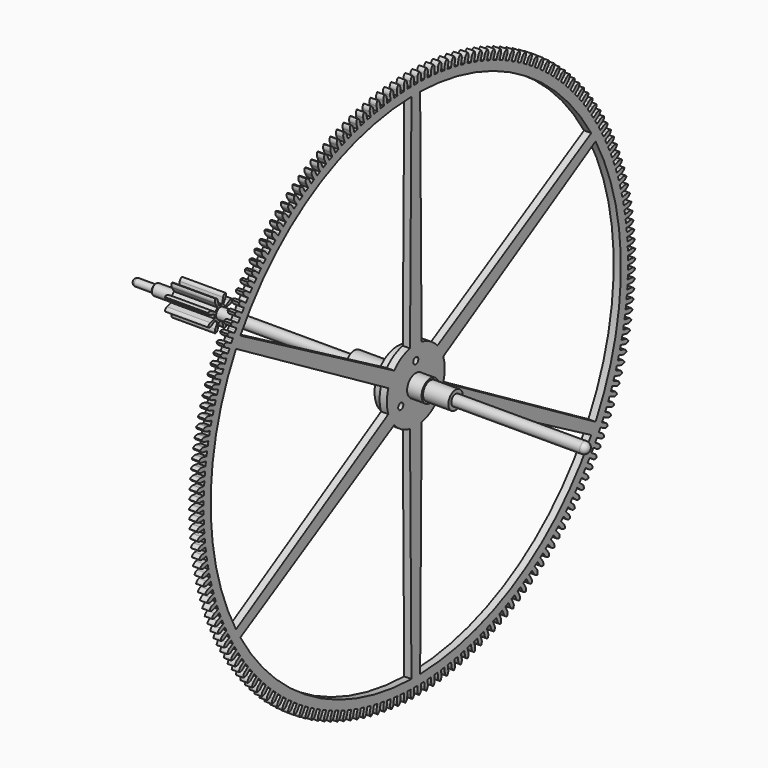
from build123d import *

# Parameters (mm, degrees)
F3_R      = 0.79375
F6_R      = 0.79375
F7_SIZE   = 0.1984375
F8_R      = 1.190625
F2_R      = 0.7
F9_DEPTH  = 2.38125
F11_R     = 1.190625
F12_DEPTH = 9.525
F13_R     = 6.35
F13_R_2   = 0.7
F13_R_3   = 2.38125
F14_DEPTH = 1.5875


with BuildPart() as f1:
    # F0 (on Front) → F1 (revolve)
    with BuildSketch(Plane.XZ):
        Polygon((-1.5875, 2.38125), (-11.1125, 2.38125), (-11.1125, 1.190625), (11.1125, 1.190625), (11.1125, 1.984375), (5.55625, 1.984375), (5.55625, 2.38125), (0.79375, 2.38125), (0.79375, 6.35), (-1.5875, 6.35), align=None)
    revolve(axis=Axis((0, 0, 0), (-1, 0, 0)))

    # F3
    f3_edges = [f1.edges().sort_by_distance(p)[0] for p in [
        (-1.5875, 0, -2.38125),
    ]]
    fillet(f3_edges, radius=F3_R)

    # F2 (on face) → F9 (cut, through all)
    with BuildSketch(Plane(origin=(-1.5875, 0, 0), x_dir=(0, -1, 0), z_dir=(-1, 0, 0))):
        with Locations((0, 4.7625)):
            Circle(F2_R)
        with Locations((4.1244459855, -2.38125)):
            Circle(F2_R)
        with Locations((-4.1244459855, -2.38125)):
            Circle(F2_R)
    extrude(amount=-F9_DEPTH, mode=Mode.SUBTRACT)


with BuildPart() as f5:
    # F4 (on Front) → F5 (revolve)
    with BuildSketch(Plane.XZ):
        Polygon((40.48125, 1.190625), (-54.76875, 1.190625), (-54.76875, 0.79375), (-59.53125, 0.79375), (-59.53125, 0), (40.48125, 0), align=None)
    revolve(axis=Axis((-9.525, 0, 0), (1, 0, 0)))

    # F6
    f6_edges = [f5.edges().sort_by_distance(p)[0] for p in [
        (-59.53125, 0, -0.79375),
    ]]
    fillet(f6_edges, radius=F6_R)

    # F7
    f7_edges = [f5.edges().sort_by_distance(p)[0] for p in [
        (-54.76875, 0, -1.190625),
    ]]
    chamfer(f7_edges, length=F7_SIZE)

    # F8
    f8_edges = [f5.edges().sort_by_distance(p)[0] for p in [
        (40.48125, 0, -1.190625),
    ]]
    fillet(f8_edges, radius=F8_R)


with BuildPart() as f12:
    # F11 (on offset) → F12 (new body)
    with BuildSketch(Plane(origin=(-50.00625, 0, 0), x_dir=(0, -1, 0), z_dir=(-1, 0, 0))):
        with BuildLine():
            Line((0.7317179963, 2.7728054793), (0.4347363988, 1.575))
            Line((0.4347363988, 1.575), (0, 1.575))
            Line((0, 1.575), (-0.4347363988, 1.575))
            Line((-0.4347363988, 1.575), (-0.7317179963, 2.7728054793))
            ThreePointArc((-0.7317179963, 2.7728054793), (-0.9713688505, 3.1705232545), (-1.3934460481, 3.3640763478))
            ThreePointArc((-1.3934460481, 3.3640763478), (-1.555036992, 2.9287599944), (-1.4432668002, 2.4780723144))
            Line((-1.4432668002, 2.4780723144), (-0.8062881248, 1.421098236))
            Line((-0.8062881248, 1.421098236), (-1.1136931804, 1.1136931804))
            Line((-1.1136931804, 1.1136931804), (-1.421098236, 0.8062881248))
            Line((-1.421098236, 0.8062881248), (-2.4780723144, 1.4432668002))
            ThreePointArc((-2.4780723144, 1.4432668002), (-2.9287599944, 1.555036992), (-3.3640763478, 1.3934460481))
            ThreePointArc((-3.3640763478, 1.3934460481), (-3.1705232545, 0.9713688505), (-2.7728054793, 0.7317179963))
            Line((-2.7728054793, 0.7317179963), (-1.575, 0.4347363988))
            Line((-1.575, 0.4347363988), (-1.575, 0))
            Line((-1.575, 0), (-1.575, -0.4347363988))
            Line((-1.575, -0.4347363988), (-2.7728054793, -0.7317179963))
            ThreePointArc((-2.7728054793, -0.7317179963), (-3.1705232545, -0.9713688505), (-3.3640763478, -1.3934460481))
            ThreePointArc((-3.3640763478, -1.3934460481), (-2.9287599944, -1.555036992), (-2.4780723144, -1.4432668002))
            Line((-2.4780723144, -1.4432668002), (-1.421098236, -0.8062881248))
            Line((-1.421098236, -0.8062881248), (-1.1136931804, -1.1136931804))
            Line((-1.1136931804, -1.1136931804), (-0.8062881248, -1.421098236))
            Line((-0.8062881248, -1.421098236), (-1.4432668002, -2.4780723144))
            ThreePointArc((-1.4432668002, -2.4780723144), (-1.555036992, -2.9287599944), (-1.3934460481, -3.3640763478))
            ThreePointArc((-1.3934460481, -3.3640763478), (-0.9713688505, -3.1705232545), (-0.7317179963, -2.7728054793))
            Line((-0.7317179963, -2.7728054793), (-0.4347363988, -1.575))
            Line((-0.4347363988, -1.575), (0, -1.575))
            Line((0, -1.575), (0.4347363988, -1.575))
            Line((0.4347363988, -1.575), (0.7317179963, -2.7728054793))
            ThreePointArc((0.7317179963, -2.7728054793), (0.9713688505, -3.1705232545), (1.3934460481, -3.3640763478))
            ThreePointArc((1.3934460481, -3.3640763478), (1.555036992, -2.9287599944), (1.4432668002, -2.4780723144))
            Line((1.4432668002, -2.4780723144), (0.8062881248, -1.421098236))
            Line((0.8062881248, -1.421098236), (1.1136931804, -1.1136931804))
            Line((1.1136931804, -1.1136931804), (1.421098236, -0.8062881248))
            Line((1.421098236, -0.8062881248), (2.4780723144, -1.4432668002))
            ThreePointArc((2.4780723144, -1.4432668002), (2.9287599944, -1.555036992), (3.3640763478, -1.3934460481))
            ThreePointArc((3.3640763478, -1.3934460481), (3.1705232545, -0.9713688505), (2.7728054793, -0.7317179963))
            Line((2.7728054793, -0.7317179963), (1.575, -0.4347363988))
            Line((1.575, -0.4347363988), (1.575, 0))
            Line((1.575, 0), (1.575, 0.4347363988))
            Line((1.575, 0.4347363988), (2.7728054793, 0.7317179963))
            ThreePointArc((2.7728054793, 0.7317179963), (3.1705232545, 0.9713688505), (3.3640763478, 1.3934460481))
            ThreePointArc((3.3640763478, 1.3934460481), (2.9287599944, 1.555036992), (2.4780723144, 1.4432668002))
            Line((2.4780723144, 1.4432668002), (1.421098236, 0.8062881248))
            Line((1.421098236, 0.8062881248), (1.1136931804, 1.1136931804))
            Line((1.1136931804, 1.1136931804), (0.8062881248, 1.421098236))
            Line((0.8062881248, 1.421098236), (1.4432668002, 2.4780723144))
            ThreePointArc((1.4432668002, 2.4780723144), (1.555036992, 2.9287599944), (1.3934460481, 3.3640763478))
            ThreePointArc((1.3934460481, 3.3640763478), (0.9713688505, 3.1705232545), (0.7317179963, 2.7728054793))
        make_face()
        Circle(F11_R, mode=Mode.SUBTRACT)
    extrude(amount=-F12_DEPTH)


with BuildPart() as f14:
    # F13 (on face) → F14 (new body)
    with BuildSketch(Plane.YZ.offset(0.79375)):
        with BuildLine():
            Line((0.4648274447, 59.2724425416), (0.466529051, 58.2))
            Line((0.466529051, 58.2), (0, 58.2))
            Line((0, 58.2), (-0.466529051, 58.2))
            Line((-0.466529051, 58.2), (-0.4648274447, 59.2724425416))
            ThreePointArc((-0.4648274447, 59.2724425416), (-0.5943871725, 59.8065181935), (-0.9555800296, 60.2207189238))
            ThreePointArc((-0.9555800296, 60.2207189238), (-1.3034493082, 59.795266823), (-1.4159986914, 59.2573493932))
            Line((-1.4159986914, 59.2573493932), (-1.3802715562, 58.1855007694))
            Line((-1.3802715562, 58.1855007694), (-1.8465657296, 58.1706987667))
            Line((-1.8465657296, 58.1706987667), (-2.312859903, 58.155896764))
            Line((-2.312859903, 58.155896764), (-2.345185539, 59.2278533647))
            ThreePointArc((-2.345185539, 59.2278533647), (-2.4916251558, 59.7575494697), (-2.8657779008, 60.1600817645))
            ThreePointArc((-2.8657779008, 60.1600817645), (-3.199973326, 59.7238066875), (-3.2953990369, 59.182589117))
            Line((-3.2953990369, 59.182589117), (-3.2256823469, 58.1124136717))
            Line((-3.2256823469, 58.1124136717), (-3.691272124, 58.0828245707))
            Line((-3.691272124, 58.0828245707), (-4.1568619011, 58.0532354696))
            Line((-4.1568619011, 58.0532354696), (-4.2231822303, 59.12362676))
            ThreePointArc((-4.2231822303, 59.12362676), (-4.3863542837, 59.648409959), (-4.7730901766, 60.0388685025))
            ThreePointArc((-4.7730901766, 60.0388685025), (-5.0932752419, 59.5922097413), (-5.1714811949, 59.0482369902))
            Line((-5.1714811949, 59.0482369902), (-5.067845149, 57.9808122994))
            Line((-5.067845149, 57.9808122994), (-5.5322617203, 57.9364658938))
            Line((-5.5322617203, 57.9364658938), (-5.9966782916, 57.8921194881))
            Line((-5.9966782916, 57.8921194881), (-6.096926535, 58.9598676748))
            ThreePointArc((-6.096926535, 58.9598676748), (-6.2766667247, 59.4792095557), (-6.6755963551, 59.8572011891))
            ThreePointArc((-6.6755963551, 59.8572011891), (-6.9814486613, 59.4006084912), (-7.0423561097, 58.8544282941))
            Line((-7.0423561097, 58.8544282941), (-6.9049050605, 57.790829164))
            Line((-6.9049050605, 57.790829164), (-7.367680798, 57.7317701068))
            Line((-7.367680798, 57.7317701068), (-7.8304565354, 57.6727110495))
            Line((-7.8304565354, 57.6727110495), (-7.9645317516, 58.7367410007))
            ThreePointArc((-7.9645317516, 58.7367410007), (-8.1606590943, 59.2501186301), (-8.571380774, 59.615262748))
            ThreePointArc((-8.571380774, 59.615262748), (-8.8625923538, 59.1491958636), (-8.9061399689, 58.6013581776))
            Line((-8.9061399689, 58.6013581776), (-8.735012318, 57.5426555623))
            Line((-8.735012318, 57.5426555623), (-9.1956812456, 57.468943321))
            Line((-9.1956812456, 57.468943321), (-9.6563501733, 57.3952310796))
            Line((-9.6563501733, 57.3952310796), (-9.8241173598, 58.4544714073))
            ThreePointArc((-9.8241173598, 58.4544714073), (-10.036434372, 58.9613678576), (-10.458534539, 59.3132967907))
            ThreePointArc((-10.458534539, 59.3132967907), (-10.734812167, 58.8382250096), (-10.7609561, 58.2892814608))
            Line((-10.7609561, 58.2892814608), (-10.5563241585, 57.2365413841))
            Line((-10.5563241585, 57.2365413841), (-11.0144224218, 57.1482501807))
            Line((-11.0144224218, 57.1482501807), (-11.472520685, 57.0599589773))
            Line((-11.472520685, 57.0599589773), (-11.6738109145, 58.1133431161))
            ThreePointArc((-11.6738109145, 58.1133431161), (-11.902103811, 58.6132479855), (-12.3351574462, 58.9516073714))
            ThreePointArc((-12.3351574462, 58.9516073714), (-12.5962229343, 58.4680090505), (-12.6049368606, 57.9185123785))
            Line((-12.6049368606, 57.9185123785), (-12.3670066754, 56.8727948605))
            Line((-12.3670066754, 56.8727948605), (-12.8220730082, 56.7700135967))
            Line((-12.8220730082, 56.7700135967), (-13.277139341, 56.6672323329))
            Line((-13.277139341, 56.6672323329), (-13.5117499312, 57.7136996145))
            ThreePointArc((-13.5117499312, 57.7136996145), (-13.7557888403, 58.2061095412), (-14.1993598955, 58.5305586805))
            ThreePointArc((-14.1993598955, 58.5305586805), (-14.4449503728, 58.0389207624), (-14.4362255182, 57.4894242639))
            Line((-14.4362255182, 57.4894242639), (-14.1652366649, 56.4517822534))
            Line((-14.1652366649, 56.4517822534), (-14.6168128539, 56.3346144213))
            Line((-14.6168128539, 56.3346144213), (-15.068389043, 56.2174465892))
            Line((-15.068389043, 56.2174465892), (-15.3360837611, 57.2559433096))
            ThreePointArc((-15.3360837611, 57.2559433096), (-15.5956229564, 57.7403624784), (-16.0492647931, 58.0505746784))
            ThreePointArc((-16.0492647931, 58.0505746784), (-16.2791329708, 57.5513922009), (-16.2529781203, 57.0024491721))
            Line((-16.2529781203, 57.0024491721), (-15.9492034618, 55.9739274867))
            Line((-15.9492034618, 55.9739274867), (-16.3968348082, 55.8424910644))
            Line((-16.3968348082, 55.8424910644), (-16.8444661546, 55.711054642))
            Line((-16.8444661546, 55.711054642), (-17.1449754546, 56.7405351232))
            ThreePointArc((-17.1449754546, 56.7405351232), (-17.4197536021, 57.2164757651), (-17.8830094414, 57.5121386684))
            ThreePointArc((-17.8830094414, 57.5121386684), (-18.0969238618, 57.0059142658), (-18.0533653513, 56.458077446))
            Line((-18.0533653513, 56.458077446), (-17.7171107627, 55.4397117198))
            Line((-17.7171107627, 55.4397117198), (-18.1603465397, 55.2941390525))
            Line((-18.1603465397, 55.2941390525), (-18.6035823166, 55.1485663852))
            Line((-18.6035823166, 55.1485663852), (-18.9366036112, 56.1679940275))
            ThreePointArc((-18.9366036112, 56.1679940275), (-19.2263440325, 56.6349769108), (-19.6987474151, 56.9157928098))
            ThreePointArc((-19.6987474151, 56.9157928098), (-19.8964926844, 56.4030362073), (-19.8355743736, 55.8568572216))
            Line((-19.8355743736, 55.8568572216), (-19.467178435, 54.8496728626))
            Line((-19.467178435, 54.8496728626), (-19.9055723416, 54.6901105297))
            Line((-19.9055723416, 54.6901105297), (-20.3439662481, 54.5305481969))
            Line((-20.3439662481, 54.5305481969), (-20.7091642131, 55.538896523))
            ThreePointArc((-20.7091642131, 55.538896523), (-21.0135751643, 55.9964514354), (-21.4946504199, 56.2621375724))
            ThreePointArc((-21.4946504199, 56.2621375724), (-21.6760274255, 55.7433650723), (-21.597810654, 55.1993938767))
            Line((-21.597810654, 55.1993938767), (-21.1976443087, 54.2044050343))
            Line((-21.1976443087, 54.2044050343), (-21.6307549194, 54.0310137015))
            Line((-21.6307549194, 54.0310137015), (-22.0638655302, 53.8576223688))
            Line((-22.0638655302, 53.8576223688), (-22.4608724421, 54.8538760576))
            ThreePointArc((-22.4608724421, 54.8538760576), (-22.7796474071, 55.30154228), (-23.2689101338, 55.5518311316))
            ThreePointArc((-23.2689101338, 55.5518311316), (-23.4337362444, 55.0275650939), (-23.3382997697, 54.4863494213))
            Line((-23.3382997697, 54.4863494213), (-22.9067659514, 53.5045579647))
            Line((-22.9067659514, 53.5045579647), (-23.3341571607, 53.3175122225))
            Line((-23.3341571607, 53.3175122225), (-23.7615483699, 53.1304664804))
            Line((-23.7615483699, 53.1304664804), (-24.1899644764, 54.1136223887))
            ThreePointArc((-24.1899644764, 54.1136223887), (-24.5227824759, 54.5509491593), (-25.0197400276, 54.7855887058))
            ThreePointArc((-25.0197400276, 54.7855887058), (-25.1678492772, 54.256357022), (-25.0552891959, 53.7184418306))
            Line((-25.0552891959, 53.7184418306), (-24.5928224226, 52.7508363407))
            Line((-24.5928224226, 52.7508363407), (-25.0140638836, 52.5503245283))
            Line((-25.0140638836, 52.5503245283), (-25.4353053446, 52.3498127158))
            Line((-25.4353053446, 52.3498127158), (-25.894699267, 53.3188808892))
            ThreePointArc((-25.894699267, 53.3188808892), (-26.2412251814, 53.7454278569), (-26.745377164, 53.9641818362))
            ThreePointArc((-26.745377164, 53.9641818362), (-26.8766204193, 53.4305173976), (-26.7470500698, 52.8964443225))
            Line((-26.7470500698, 52.8964443225), (-26.2541160062, 51.943999096))
            Line((-26.2541160062, 51.943999096), (-26.6687835645, 51.7302231117))
            Line((-26.6687835645, 51.7302231117), (-27.0834511229, 51.5164471274))
            Line((-27.0834511229, 51.5164471274), (-27.5733602905, 52.4704517962))
            ThreePointArc((-27.5733602905, 52.4704517962), (-27.9332451976, 52.8857894644), (-28.4440839727, 53.0884376097))
            ThreePointArc((-28.4440839727, 53.0884376097), (-28.5583290828, 52.5508777714), (-28.4118789314, 52.0211845789))
            Line((-28.4118789314, 52.0211845789), (-27.8889739205, 51.0848586473))
            Line((-27.8889739205, 51.0848586473), (-28.296650041, 50.8580337455))
            Line((-28.296650041, 50.8580337455), (-28.7043261616, 50.6312088436))
            Line((-28.7043261616, 50.6312088436), (-29.2242572774, 51.5691894059))
            ThreePointArc((-29.2242572774, 51.5691894059), (-29.5971388037, 51.9728995648), (-30.11415, 52.1592378268))
            ThreePointArc((-30.11415, 52.1592378268), (-30.2112819297, 51.6183238657), (-30.0480994394, 51.093543912))
            Line((-30.0480994394, 51.093543912), (-29.495750002, 50.1742800763))
            Line((-29.495750002, 50.1742800763), (-29.8960241896, 49.9346346503))
            Line((-29.8960241896, 49.9346346503), (-30.2962983771, 49.6949892243))
            Line((-30.2962983771, 49.6949892243), (-30.8457279145, 50.6160012133))
            ThreePointArc((-30.8457279145, 50.6160012133), (-31.2312305998, 51.007677361), (-31.7538936309, 51.1775181126))
            ThreePointArc((-31.7538936309, 51.1775181126), (-31.8338145765, 50.6337946834), (-31.6540640583, 50.1144563773))
            Line((-31.6540640583, 50.1144563773), (-31.0728263636, 49.2131802583))
            Line((-31.0728263636, 49.2131802583), (-31.4652955759, 48.9609556108))
            Line((-31.4652955759, 48.9609556108), (-31.8577647882, 48.7087309633))
            Line((-31.8577647882, 48.7087309633), (-32.4361395183, 49.611846998))
            ThreePointArc((-32.4361395183, 49.611846998), (-32.8338751941, 49.9910947498), (-33.3616637825, 50.1442669759))
            ThreePointArc((-33.3616637825, 50.1442669759), (-33.4242932706, 49.598281562), (-33.2281557178, 49.0849078332))
            Line((-33.2281557178, 49.0849078332), (-32.618615023, 48.2025269394))
            Line((-32.618615023, 48.2025269394), (-33.0028840768, 47.9379770392))
            Line((-33.0028840768, 47.9379770392), (-33.3871531307, 47.6734271391))
            Line((-33.3871531307, 47.6734271391), (-33.9938906791, 48.5577378582))
            ThreePointArc((-33.9938906791, 48.5577378582), (-34.4034588592, 48.9241753437), (-34.9358415667, 49.0605248129))
            ThreePointArc((-34.9358415667, 49.0605248129), (-34.9811165346, 48.5128271752), (-34.7687894413, 48.0059349476))
            Line((-34.7687894413, 48.0059349476), (-34.1315595019, 47.1433377618))
            Line((-34.1315595019, 47.1433377618), (-34.507241471, 46.8667289883))
            Line((-34.507241471, 46.8667289883), (-34.88292344, 46.5901202148))
            Line((-34.88292344, 46.5901202148), (-35.5174128735, 47.4547351924))
            ThreePointArc((-35.5174128735, 47.4547351924), (-35.9384011576, 47.8079934402), (-36.4748419198, 47.92738286))
            ThreePointArc((-36.4748419198, 47.92738286), (-36.5027167794, 47.3785244838), (-36.2744139409, 46.8786241548))
            Line((-36.2744139409, 46.8786241548), (-35.6101363937, 46.0366792392))
            Line((-35.6101363937, 46.0366792392), (-35.976852998, 45.748290114))
            Line((-35.976852998, 45.748290114), (-36.3435696024, 45.4599009888))
            Line((-36.3435696024, 45.4599009888), (-37.0051720438, 46.3039496308))
            ThreePointArc((-37.0051720438, 46.3039496308), (-37.4371565323, 46.6436729398), (-37.977115199, 46.7459820953))
            ThreePointArc((-37.977115199, 46.7459820953), (-37.9875618827, 46.1965156343), (-37.7435131806, 45.7041105612))
            Line((-37.7435131806, 45.7041105612), (-37.0528568967, 44.8836656831))
            Line((-37.0528568967, 44.8836656831), (-37.4102388838, 44.5837865895))
            Line((-37.4102388838, 44.5837865895), (-37.7676208708, 44.283907496))
            Line((-37.7676208708, 44.283907496), (-38.4556701426, 45.106539917))
            ThreePointArc((-38.4556701426, 45.106539917), (-38.8982158638, 45.4323862146), (-39.4411487423, 45.5175120891))
            ThreePointArc((-39.4411487423, 45.5175120891), (-39.4341567312, 44.9679908094), (-39.1746079019, 44.4835768024))
            Line((-39.1746079019, 44.4835768024), (-38.4582683136, 43.6854580802))
            Line((-38.4582683136, 43.6854580802), (-38.80595583, 43.3743909711))
            Line((-38.80595583, 43.3743909711), (-39.1536433465, 43.0633238621))
            Line((-39.1536433465, 43.0633238621), (-39.8674466414, 43.863711741))
            ThreePointArc((-39.8674466414, 43.863711741), (-40.3201079893, 44.1753529275), (-40.8654683921, 44.2432098065))
            ThreePointArc((-40.8654683921, 44.2432098065), (-40.8410447266, 43.6941870296), (-40.5662571137, 43.2182518525))
            Line((-40.5662571137, 43.2182518525), (-39.8249555143, 42.443262924))
            Line((-39.8249555143, 42.443262924), (-40.1625984683, 42.1213210177))
            Line((-40.1625984683, 42.1213210177), (-40.5002414222, 41.7993791114))
            Line((-40.5002414222, 41.7993791114), (-41.2390800008, 42.5767165254))
            ThreePointArc((-41.2390800008, 42.5767165254), (-41.7014011837, 42.8738388047), (-42.2486399792, 42.9243583621))
            ThreePointArc((-42.2486399792, 42.9243583621), (-42.2068092519, 42.3763869073), (-41.9170595432, 41.9094097865))
            Line((-41.9170595432, 41.9094097865), (-41.1515423606, 41.158331))
            Line((-41.1515423606, 41.158331), (-41.4788007742, 40.8258384645))
            Line((-41.4788007742, 40.8258384645), (-41.8060591879, 40.4933459291))
            Line((-41.8060591879, 40.4933459291), (-42.5691891024, 41.2468501654))
            ThreePointArc((-42.5691891024, 41.2468501654), (-43.0407046021, 41.5291543605), (-43.5892707672, 41.5622857272))
            ThreePointArc((-43.5892707672, 41.5622857272), (-43.5300750979, 41.0159173554), (-43.225655047, 40.5583684973))
            Line((-43.225655047, 40.5583684973), (-42.436693092, 39.8319561253))
            Line((-42.436693092, 39.8319561253), (-42.7532374439, 39.4892477526))
            Line((-42.7532374439, 39.4892477526), (-43.0697817957, 39.1465393799))
            Line((-43.0697817957, 39.1465393799), (-43.8564346389, 39.8754517236))
            ThreePointArc((-43.8564346389, 39.8754517236), (-44.3366696793, 40.1426535781), (-44.8860108544, 40.1583633938))
            ThreePointArc((-44.8860108544, 40.1583633938), (-44.8095098483, 39.6141482515), (-44.4907259802, 39.166488369))
            Line((-44.4907259802, 39.166488369), (-43.6791136707, 38.4654738473))
            Line((-43.6791136707, 38.4654738473), (-43.9846252274, 38.1128947156))
            Line((-43.9846252274, 38.1128947156), (-44.2901367842, 37.7603155839))
            Line((-44.2901367842, 37.7603155839), (-45.0995204634, 38.463902082))
            ThreePointArc((-45.0995204634, 38.463902082), (-45.5879914884, 38.7157325463), (-46.1375545335, 38.7140049925))
            ThreePointArc((-46.1375545335, 38.7140049925), (-46.0438252206, 38.1724910583), (-45.7109985236, 37.7351709069))
            Line((-45.7109985236, 37.7351709069), (-44.8775530844, 37.0602600977))
            Line((-44.8775530844, 37.0602600977), (-45.1717242218, 36.6981652243))
            Line((-45.1717242218, 36.6981652243), (-45.4658953592, 36.3360703509))
            Line((-45.4658953592, 36.3360703509), (-46.2971948936, 37.0136225515))
            ThreePointArc((-46.2971948936, 37.0136225515), (-46.7934100544, 37.2498280536), (-47.3426416061, 37.2306648698))
            ThreePointArc((-47.3426416061, 37.2306648698), (-47.2317783638, 36.6923974023), (-46.8852439663, 36.2658573264))
            Line((-46.8852439663, 36.2658573264), (-46.0308046063, 35.6177298077))
            Line((-46.0308046063, 35.6177298077), (-46.3133391189, 35.2464837914))
            Line((-46.3133391189, 35.2464837914), (-46.5958736315, 34.8752377751))
            Line((-46.5958736315, 34.8752377751), (-47.448251973, 35.5260734406))
            ThreePointArc((-47.448251973, 35.5260734406), (-47.951711623, 35.7464161416), (-48.5000586517, 35.7098366235))
            ThreePointArc((-48.5000586517, 35.7098366235), (-48.3721731099, 35.1753576125), (-48.0122799426, 34.7600271017))
            Line((-48.0122799426, 34.7600271017), (-47.1377070098, 34.1393354829))
            Line((-47.1377070098, 34.1393354829), (-47.4083204093, 33.759312137))
            Line((-47.4083204093, 33.759312137), (-47.6789338089, 33.3792887912))
            Line((-47.6789338089, 33.3792887912), (-48.5515326847, 34.0027525851))
            ThreePointArc((-48.5515326847, 34.0027525851), (-49.0617298827, 34.2070106186), (-49.6086402493, 34.1530515987))
            ThreePointArc((-49.6086402493, 34.1530515987), (-49.463861178, 33.6228992192), (-49.0909716229, 33.2191964762))
            Line((-49.0909716229, 33.2191964762), (-48.197145738, 32.6265657412))
            Line((-48.197145738, 32.6265657412), (-48.4555655397, 32.238147717))
            Line((-48.4555655397, 32.238147717), (-48.7139853415, 31.8497296928))
            Line((-48.7139853415, 31.8497296928), (-49.6059261186, 32.4451938401))
            ThreePointArc((-49.6059261186, 32.4451938401), (-50.1223471391, 32.6331615355), (-50.6672701514, 32.561877346))
            ThreePointArc((-50.6672701514, 32.561877346), (-50.5057433308, 32.0365854164), (-50.1202328559, 31.6449169357))
            Line((-50.1202328559, 31.6449169357), (-49.208054026, 31.0809438134))
            Line((-49.208054026, 31.0809438134), (-49.4540200231, 30.6845222149))
            Line((-49.4540200231, 30.6845222149), (-49.6999860201, 30.2881006165))
            Line((-49.6999860201, 30.2881006165), (-50.6103705897, 30.8549655351))
            ThreePointArc((-50.6103705897, 30.8549655351), (-51.1324954407, 31.026453625), (-51.6748824073, 30.9379160429))
            ThreePointArc((-51.6748824073, 30.9379160429), (-51.4967704812, 30.4180134878), (-51.099027263, 30.0387736463))
            Line((-51.099027263, 30.0387736463), (-50.1694139748, 29.5040260098))
            Line((-50.1694139748, 29.5040260098), (-50.4026785003, 29.1))
            Line((-50.4026785003, 29.1), (-50.6359430257, 28.6959739902))
            Line((-50.6359430257, 28.6959739902), (-51.5638547077, 29.2336688953))
            ThreePointArc((-51.5638547077, 29.2336688953), (-52.0911576537, 29.3885047057), (-52.630462437, 29.2828028809))
            ThreePointArc((-52.630462437, 29.2828028809), (-52.4359447489, 28.7688131981), (-52.0263692812, 28.4023838581))
            Line((-52.0263692812, 28.4023838581), (-51.0802575763, 27.8974001529))
            Line((-51.0802575763, 27.8974001529), (-51.3005857526, 27.4861765518))
            Line((-51.3005857526, 27.4861765518), (-51.520913929, 27.0749529506))
            Line((-51.520913929, 27.0749529506), (-52.465418395, 27.582936429))
            ThreePointArc((-52.465418395, 27.582936429), (-52.9973684865, 27.7209640532), (-53.5330480522, 27.5982044186))
            ThreePointArc((-53.5330480522, 27.5982044186), (-53.3223204651, 27.090645152), (-52.9013251555, 26.7373952769))
            Line((-52.9013251555, 26.7373952769), (-51.9396676884, 26.2626839789))
            Line((-51.9396676884, 26.2626839789), (-52.1468376638, 25.8446768537))
            Line((-52.1468376638, 25.8446768537), (-52.3540076391, 25.4266697284))
            Line((-52.3540076391, 25.4266697284), (-53.3141538531, 25.9044302837))
            ThreePointArc((-53.3141538531, 25.9044302837), (-53.8502154617, 26.0255107398), (-54.3817304259, 25.8858169038))
            ThreePointArc((-54.3817304259, 25.8858169038), (-54.1550051245, 25.3851991227), (-53.7230138797, 25.0454844051))
            Line((-53.7230138797, 25.0454844051), (-52.7467789579, 24.6015235082))
            Line((-52.7467789579, 24.6015235082), (-52.9405821296, 24.1771537567))
            Line((-52.9405821296, 24.1771537567), (-53.1343853014, 23.7527840052))
            Line((-53.1343853014, 23.7527840052), (-54.1092064776, 24.1998405731))
            ThreePointArc((-54.1092064776, 24.1998405731), (-54.6488398346, 24.3038519432), (-55.1756550068, 24.1473645656))
            ThreePointArc((-55.1756550068, 24.1473645656), (-54.9331602843, 23.6541923497), (-54.4906080828, 23.3283548535))
            Line((-54.4906080828, 23.3283548535), (-53.500778692, 22.9155913888))
            Line((-53.500778692, 22.9155913888), (-53.6810199169, 22.4852863153))
            Line((-53.6810199169, 22.4852863153), (-53.8612611417, 22.0549812418))
            Line((-53.8612611417, 22.0549812418), (-54.8497757179, 22.4708836742))
            ThreePointArc((-54.8497757179, 22.4708836742), (-55.3924374581, 22.5577212278), (-55.9140223801, 22.3845978782))
            ThreePointArc((-55.9140223801, 22.3845978782), (-55.6560024082, 21.89936781), (-55.2033348625, 21.5877356261))
            Line((-55.2033348625, 21.5877356261), (-54.2009076772, 21.2065852114))
            Line((-54.2009076772, 21.2065852114), (-54.3674054674, 20.7707780966))
            Line((-54.3674054674, 20.7707780966), (-54.5339032577, 20.3349709819))
            Line((-54.5339032577, 20.3349709819), (-55.5351158834, 20.7193005003))
            ThreePointArc((-55.5351158834, 20.7193005003), (-56.0802595925, 20.7888767993), (-56.5960890725, 20.5992917983))
            ThreePointArc((-56.5960890725, 20.5992917983), (-56.3228036554, 20.1224924633), (-55.8604765634, 19.8253793787))
            Line((-55.8604765634, 19.8253793787), (-54.8464609427, 19.4762258002))
            Line((-54.8464609427, 19.4762258002), (-54.9990476492, 19.0353554651))
            Line((-54.9990476492, 19.0353554651), (-55.1516343557, 18.5944851299))
            Line((-55.1516343557, 18.5944851299), (-56.1645368947, 18.9468547471))
            ThreePointArc((-56.1645368947, 18.9468547471), (-56.7116136593, 18.999099734), (-57.2211683006, 18.7932439776))
            ThreePointArc((-57.2211683006, 18.7932439776), (-56.9328926136, 18.3253554724), (-56.4613714995, 18.0430606549))
            Line((-56.4613714995, 18.0430606549), (-55.4367884711, 17.7262554806))
            Line((-55.4367884711, 17.7262554806), (-55.575310452, 17.2807658441))
            Line((-55.575310452, 17.2807658441), (-55.713832433, 16.8352762076))
            Line((-55.713832433, 16.8352762076), (-56.7374049782, 17.1553311172))
            ThreePointArc((-56.7374049782, 17.1553311172), (-57.2858639383, 17.1901921858), (-57.7886306627, 16.9682729532))
            ThreePointArc((-57.7886306627, 16.9682729532), (-57.4856549749, 16.5097664019), (-57.0054146205, 16.2425740984))
            Line((-57.0054146205, 16.2425740984), (-55.9712958528, 15.9584363243))
            Line((-55.9712958528, 15.9584363243), (-56.0956136282, 15.5087759568))
            Line((-56.0956136282, 15.5087759568), (-56.2199314036, 15.0591155892))
            Line((-56.2199314036, 15.0591155892), (-57.2531433043, 15.3465335231))
            ThreePointArc((-57.2531433043, 15.3465335231), (-57.8024322082, 15.3639755712), (-58.2979047723, 15.1262163163))
            ThreePointArc((-58.2979047723, 15.1262163163), (-57.9805341545, 14.6775533961), (-57.4920581212, 14.4257326467))
            Line((-57.4920581212, 14.4257326467), (-56.449444884, 14.1745483754))
            Line((-56.449444884, 14.1745483754), (-56.5594332764, 13.7211700466))
            Line((-56.5594332764, 13.7211700466), (-56.6694216689, 13.2677917179))
            Line((-56.6694216689, 13.2677917179), (-57.7112325683, 13.5222832706))
            ThreePointArc((-57.7112325683, 13.5222832706), (-58.2607983287, 13.5222887355), (-58.7484778335, 13.2689288618))
            ThreePointArc((-58.7484778335, 13.2689288618), (-58.417031851, 12.8305613383), (-57.9208119927, 12.594365705))
            Line((-57.9208119927, 12.594365705), (-56.8707541092, 12.3763878577))
            Line((-56.8707541092, 12.3763878577), (-56.9663023697, 11.9197480814))
            Line((-56.9663023697, 11.9197480814), (-57.0618506302, 11.4631083051))
            Line((-57.0618506302, 11.4631083051), (-58.111211513, 11.6844172251))
            ThreePointArc((-58.111211513, 11.6844172251), (-58.6605007637, 11.6669861013), (-59.1398961573, 11.3982807207))
            ThreePointArc((-59.1398961573, 11.3982807207), (-58.7947085483, 10.9706499927), (-58.2912445162, 10.7503173046))
            Line((-58.2912445162, 10.7503173046), (-57.2347993058, 10.5657653666))
            Line((-57.2347993058, 10.5657653666), (-57.3158112253, 10.1063239402))
            Line((-57.3158112253, 10.1063239402), (-57.3968231448, 9.6468825138))
            Line((-57.3968231448, 9.6468825138), (-58.4526773937, 9.8347859619))
            ThreePointArc((-58.4526773937, 9.8347859619), (-59.0011370469, 9.7999358011), (-59.4717656189, 9.5161554771))
            ThreePointArc((-59.4717656189, 9.5161554771), (-59.1131839578, 9.0996921325), (-58.6029826977, 8.8954442459))
            Line((-58.6029826977, 8.8954442459), (-57.541213911, 8.7445040454))
            Line((-57.541213911, 8.7445040454), (-57.6076079175, 8.2827235875))
            Line((-57.6076079175, 8.2827235875), (-57.6740019239, 7.8209431296))
            Line((-57.6740019239, 7.8209431296), (-58.735286383, 7.9752519028))
            ThreePointArc((-58.735286383, 7.9752519028), (-59.2823641865, 7.9230177962), (-59.7437520536, 7.6244482716))
            ThreePointArc((-59.7437520536, 7.6244482716), (-59.3721374019, 7.2195716538), (-58.8557126432, 7.0316142289))
            Line((-58.8557126432, 7.0316142289), (-57.7896893914, 6.9144377499))
            Line((-57.7896893914, 6.9144377499), (-57.8413986316, 6.4507832342))
            Line((-57.8413986316, 6.4507832342), (-57.8931078719, 5.9871287186))
            Line((-57.8931078719, 5.9871287186), (-58.9587539177, 6.1076874412))
            ThreePointArc((-58.9587539177, 6.1076874412), (-59.5038990104, 6.0381219841), (-59.9555815943, 5.7250638929))
            ThreePointArc((-59.9555815943, 5.7250638929), (-59.5713081365, 5.3321816783), (-59.049179875, 5.1607039725))
            Line((-59.049179875, 5.1607039725), (-57.9799755532, 5.0774092017))
            Line((-57.9799755532, 5.0774092017), (-58.0169479604, 4.6123474891))
            Line((-58.0169479604, 4.6123474891), (-58.0539203676, 4.1472857765))
            Line((-58.0539203676, 4.1472857765), (-59.1228549849, 4.233973056))
            ThreePointArc((-59.1228549849, 4.233973056), (-59.665518452, 4.1471462949), (-60.1070409466, 3.8199148603))
            ThreePointArc((-60.1070409466, 3.8199148603), (-59.7104956133, 3.4394226479), (-59.1831895881, 3.2845973246))
            Line((-59.1831895881, 3.2845973246), (-58.1118807944, 3.2352681328))
            Line((-58.1118807944, 3.2352681328), (-58.1340791405, 2.7692675009))
            Line((-58.1340791405, 2.7692675009), (-58.1562774865, 2.3032668691))
            Line((-58.1562774865, 2.3032668691), (-59.2274243488, 2.3559954188))
            ThreePointArc((-59.2274243488, 2.3559954188), (-59.7670597741, 2.2519947809), (-60.1979776036, 1.9109194971))
            ThreePointArc((-60.1979776036, 1.9109194971), (-59.7895596825, 1.5432004104), (-59.257606846, 1.4051833656))
            Line((-59.257606846, 1.4051833656), (-58.1852722976, 1.3898694231))
            Line((-58.1852722976, 1.3898694231), (-58.1926742306, 0.9233990952))
            Line((-58.1926742306, 0.9233990952), (-58.2000761637, 0.4569287673))
            Line((-58.2000761637, 0.4569287673), (-59.2723567168, 0.475645494))
            ThreePointArc((-59.2723567168, 0.475645494), (-59.8084207333, 0.3545756991), (-60.2283, 0))
            ThreePointArc((-60.2283, 0), (-59.8084207333, -0.3545756991), (-59.2723567168, -0.475645494))
            Line((-59.2723567168, -0.475645494), (-58.2000761637, -0.4569287673))
            Line((-58.2000761637, -0.4569287673), (-58.1926742306, -0.9233990952))
            Line((-58.1926742306, -0.9233990952), (-58.1852722976, -1.3898694231))
            Line((-58.1852722976, -1.3898694231), (-59.257606846, -1.4051833656))
            ThreePointArc((-59.257606846, -1.4051833656), (-59.7895596825, -1.5432004104), (-60.1979776036, -1.9109194971))
            ThreePointArc((-60.1979776036, -1.9109194971), (-59.7670597741, -2.2519947809), (-59.2274243488, -2.3559954188))
            Line((-59.2274243488, -2.3559954188), (-58.1562774865, -2.3032668691))
            Line((-58.1562774865, -2.3032668691), (-58.1340791405, -2.7692675009))
            Line((-58.1340791405, -2.7692675009), (-58.1118807944, -3.2352681328))
            Line((-58.1118807944, -3.2352681328), (-59.1831895881, -3.2845973246))
            ThreePointArc((-59.1831895881, -3.2845973246), (-59.7104956133, -3.4394226479), (-60.1070409466, -3.8199148603))
            ThreePointArc((-60.1070409466, -3.8199148603), (-59.665518452, -4.1471462949), (-59.1228549849, -4.233973056))
            Line((-59.1228549849, -4.233973056), (-58.0539203676, -4.1472857765))
            Line((-58.0539203676, -4.1472857765), (-58.0169479604, -4.6123474891))
            Line((-58.0169479604, -4.6123474891), (-57.9799755532, -5.0774092017))
            Line((-57.9799755532, -5.0774092017), (-59.049179875, -5.1607039725))
            ThreePointArc((-59.049179875, -5.1607039725), (-59.5713081365, -5.3321816783), (-59.9555815943, -5.7250638929))
            ThreePointArc((-59.9555815943, -5.7250638929), (-59.5038990104, -6.0381219841), (-58.9587539177, -6.1076874412))
            Line((-58.9587539177, -6.1076874412), (-57.8931078719, -5.9871287186))
            Line((-57.8931078719, -5.9871287186), (-57.8413986316, -6.4507832342))
            Line((-57.8413986316, -6.4507832342), (-57.7896893914, -6.9144377499))
            Line((-57.7896893914, -6.9144377499), (-58.8557126432, -7.0316142289))
            ThreePointArc((-58.8557126432, -7.0316142289), (-59.3721374019, -7.2195716538), (-59.7437520536, -7.6244482716))
            ThreePointArc((-59.7437520536, -7.6244482716), (-59.2823641865, -7.9230177962), (-58.735286383, -7.9752519028))
            Line((-58.735286383, -7.9752519028), (-57.6740019239, -7.8209431296))
            Line((-57.6740019239, -7.8209431296), (-57.6076079175, -8.2827235875))
            Line((-57.6076079175, -8.2827235875), (-57.541213911, -8.7445040454))
            Line((-57.541213911, -8.7445040454), (-58.6029826977, -8.8954442459))
            ThreePointArc((-58.6029826977, -8.8954442459), (-59.1131839578, -9.0996921325), (-59.4717656189, -9.5161554771))
            ThreePointArc((-59.4717656189, -9.5161554771), (-59.0011370469, -9.7999358011), (-58.4526773937, -9.8347859619))
            Line((-58.4526773937, -9.8347859619), (-57.3968231448, -9.6468825138))
            Line((-57.3968231448, -9.6468825138), (-57.3158112253, -10.1063239402))
            Line((-57.3158112253, -10.1063239402), (-57.2347993058, -10.5657653666))
            Line((-57.2347993058, -10.5657653666), (-58.2912445162, -10.7503173046))
            ThreePointArc((-58.2912445162, -10.7503173046), (-58.7947085483, -10.9706499927), (-59.1398961573, -11.3982807207))
            ThreePointArc((-59.1398961573, -11.3982807207), (-58.6605007637, -11.6669861013), (-58.111211513, -11.6844172251))
            Line((-58.111211513, -11.6844172251), (-57.0618506302, -11.4631083051))
            Line((-57.0618506302, -11.4631083051), (-56.9663023697, -11.9197480814))
            Line((-56.9663023697, -11.9197480814), (-56.8707541092, -12.3763878577))
            Line((-56.8707541092, -12.3763878577), (-57.9208119927, -12.594365705))
            ThreePointArc((-57.9208119927, -12.594365705), (-58.417031851, -12.8305613383), (-58.7484778335, -13.2689288618))
            ThreePointArc((-58.7484778335, -13.2689288618), (-58.2607983287, -13.5222887355), (-57.7112325683, -13.5222832706))
            Line((-57.7112325683, -13.5222832706), (-56.6694216689, -13.2677917179))
            Line((-56.6694216689, -13.2677917179), (-56.5594332764, -13.7211700466))
            Line((-56.5594332764, -13.7211700466), (-56.449444884, -14.1745483754))
            Line((-56.449444884, -14.1745483754), (-57.4920581212, -14.4257326467))
            ThreePointArc((-57.4920581212, -14.4257326467), (-57.9805341545, -14.6775533961), (-58.2979047723, -15.1262163163))
            ThreePointArc((-58.2979047723, -15.1262163163), (-57.8024322082, -15.3639755712), (-57.2531433043, -15.3465335231))
            Line((-57.2531433043, -15.3465335231), (-56.2199314036, -15.0591155892))
            Line((-56.2199314036, -15.0591155892), (-56.0956136282, -15.5087759568))
            Line((-56.0956136282, -15.5087759568), (-55.9712958528, -15.9584363243))
            Line((-55.9712958528, -15.9584363243), (-57.0054146205, -16.2425740984))
            ThreePointArc((-57.0054146205, -16.2425740984), (-57.4856549749, -16.5097664019), (-57.7886306627, -16.9682729532))
            ThreePointArc((-57.7886306627, -16.9682729532), (-57.2858639383, -17.1901921858), (-56.7374049782, -17.1553311172))
            Line((-56.7374049782, -17.1553311172), (-55.713832433, -16.8352762076))
            Line((-55.713832433, -16.8352762076), (-55.575310452, -17.2807658441))
            Line((-55.575310452, -17.2807658441), (-55.4367884711, -17.7262554806))
            Line((-55.4367884711, -17.7262554806), (-56.4613714995, -18.0430606549))
            ThreePointArc((-56.4613714995, -18.0430606549), (-56.9328926136, -18.3253554724), (-57.2211683006, -18.7932439776))
            ThreePointArc((-57.2211683006, -18.7932439776), (-56.7116136593, -18.999099734), (-56.1645368947, -18.9468547471))
            Line((-56.1645368947, -18.9468547471), (-55.1516343557, -18.5944851299))
            Line((-55.1516343557, -18.5944851299), (-54.9990476492, -19.0353554651))
            Line((-54.9990476492, -19.0353554651), (-54.8464609427, -19.4762258002))
            Line((-54.8464609427, -19.4762258002), (-55.8604765634, -19.8253793787))
            ThreePointArc((-55.8604765634, -19.8253793787), (-56.3228036554, -20.1224924633), (-56.5960890725, -20.5992917983))
            ThreePointArc((-56.5960890725, -20.5992917983), (-56.0802595925, -20.7888767993), (-55.5351158834, -20.7193005003))
            Line((-55.5351158834, -20.7193005003), (-54.5339032577, -20.3349709819))
            Line((-54.5339032577, -20.3349709819), (-54.3674054674, -20.7707780966))
            Line((-54.3674054674, -20.7707780966), (-54.2009076772, -21.2065852114))
            Line((-54.2009076772, -21.2065852114), (-55.2033348625, -21.5877356261))
            ThreePointArc((-55.2033348625, -21.5877356261), (-55.6560024082, -21.89936781), (-55.9140223801, -22.3845978782))
            ThreePointArc((-55.9140223801, -22.3845978782), (-55.3924374581, -22.5577212278), (-54.8497757179, -22.4708836742))
            Line((-54.8497757179, -22.4708836742), (-53.8612611417, -22.0549812418))
            Line((-53.8612611417, -22.0549812418), (-53.6810199169, -22.4852863153))
            Line((-53.6810199169, -22.4852863153), (-53.500778692, -22.9155913888))
            Line((-53.500778692, -22.9155913888), (-54.4906080828, -23.3283548535))
            ThreePointArc((-54.4906080828, -23.3283548535), (-54.9331602843, -23.6541923497), (-55.1756550068, -24.1473645656))
            ThreePointArc((-55.1756550068, -24.1473645656), (-54.6488398346, -24.3038519432), (-54.1092064776, -24.1998405731))
            Line((-54.1092064776, -24.1998405731), (-53.1343853014, -23.7527840052))
            Line((-53.1343853014, -23.7527840052), (-52.9405821296, -24.1771537567))
            Line((-52.9405821296, -24.1771537567), (-52.7467789579, -24.6015235082))
            Line((-52.7467789579, -24.6015235082), (-53.7230138797, -25.0454844051))
            ThreePointArc((-53.7230138797, -25.0454844051), (-54.1550051245, -25.3851991227), (-54.3817304259, -25.8858169038))
            ThreePointArc((-54.3817304259, -25.8858169038), (-53.8502154617, -26.0255107398), (-53.3141538531, -25.9044302837))
            Line((-53.3141538531, -25.9044302837), (-52.3540076391, -25.4266697284))
            Line((-52.3540076391, -25.4266697284), (-52.1468376638, -25.8446768537))
            Line((-52.1468376638, -25.8446768537), (-51.9396676884, -26.2626839789))
            Line((-51.9396676884, -26.2626839789), (-52.9013251555, -26.7373952769))
            ThreePointArc((-52.9013251555, -26.7373952769), (-53.3223204651, -27.090645152), (-53.5330480522, -27.5982044186))
            ThreePointArc((-53.5330480522, -27.5982044186), (-52.9973684865, -27.7209640532), (-52.465418395, -27.582936429))
            Line((-52.465418395, -27.582936429), (-51.520913929, -27.0749529506))
            Line((-51.520913929, -27.0749529506), (-51.3005857526, -27.4861765518))
            Line((-51.3005857526, -27.4861765518), (-51.0802575763, -27.8974001529))
            Line((-51.0802575763, -27.8974001529), (-52.0263692812, -28.4023838581))
            ThreePointArc((-52.0263692812, -28.4023838581), (-52.4359447489, -28.7688131981), (-52.630462437, -29.2828028809))
            ThreePointArc((-52.630462437, -29.2828028809), (-52.0911576537, -29.3885047057), (-51.5638547077, -29.2336688953))
            Line((-51.5638547077, -29.2336688953), (-50.6359430257, -28.6959739902))
            Line((-50.6359430257, -28.6959739902), (-50.4026785003, -29.1))
            Line((-50.4026785003, -29.1), (-50.1694139748, -29.5040260098))
            Line((-50.1694139748, -29.5040260098), (-51.099027263, -30.0387736463))
            ThreePointArc((-51.099027263, -30.0387736463), (-51.4967704812, -30.4180134878), (-51.6748824073, -30.9379160429))
            ThreePointArc((-51.6748824073, -30.9379160429), (-51.1324954407, -31.026453625), (-50.6103705897, -30.8549655351))
            Line((-50.6103705897, -30.8549655351), (-49.6999860201, -30.2881006165))
            Line((-49.6999860201, -30.2881006165), (-49.4540200231, -30.6845222149))
            Line((-49.4540200231, -30.6845222149), (-49.208054026, -31.0809438134))
            Line((-49.208054026, -31.0809438134), (-50.1202328559, -31.6449169357))
            ThreePointArc((-50.1202328559, -31.6449169357), (-50.5057433308, -32.0365854164), (-50.6672701514, -32.561877346))
            ThreePointArc((-50.6672701514, -32.561877346), (-50.1223471391, -32.6331615355), (-49.6059261186, -32.4451938401))
            Line((-49.6059261186, -32.4451938401), (-48.7139853415, -31.8497296928))
            Line((-48.7139853415, -31.8497296928), (-48.4555655397, -32.238147717))
            Line((-48.4555655397, -32.238147717), (-48.197145738, -32.6265657412))
            Line((-48.197145738, -32.6265657412), (-49.0909716229, -33.2191964762))
            ThreePointArc((-49.0909716229, -33.2191964762), (-49.463861178, -33.6228992192), (-49.6086402493, -34.1530515987))
            ThreePointArc((-49.6086402493, -34.1530515987), (-49.0617298827, -34.2070106186), (-48.5515326847, -34.0027525851))
            Line((-48.5515326847, -34.0027525851), (-47.6789338089, -33.3792887912))
            Line((-47.6789338089, -33.3792887912), (-47.4083204093, -33.759312137))
            Line((-47.4083204093, -33.759312137), (-47.1377070098, -34.1393354829))
            Line((-47.1377070098, -34.1393354829), (-48.0122799426, -34.7600271017))
            ThreePointArc((-48.0122799426, -34.7600271017), (-48.3721731099, -35.1753576125), (-48.5000586517, -35.7098366235))
            ThreePointArc((-48.5000586517, -35.7098366235), (-47.951711623, -35.7464161416), (-47.448251973, -35.5260734406))
            Line((-47.448251973, -35.5260734406), (-46.5958736315, -34.8752377751))
            Line((-46.5958736315, -34.8752377751), (-46.3133391189, -35.2464837914))
            Line((-46.3133391189, -35.2464837914), (-46.0308046063, -35.6177298077))
            Line((-46.0308046063, -35.6177298077), (-46.8852439663, -36.2658573264))
            ThreePointArc((-46.8852439663, -36.2658573264), (-47.2317783638, -36.6923974023), (-47.3426416061, -37.2306648698))
            ThreePointArc((-47.3426416061, -37.2306648698), (-46.7934100544, -37.2498280536), (-46.2971948936, -37.0136225515))
            Line((-46.2971948936, -37.0136225515), (-45.4658953592, -36.3360703509))
            Line((-45.4658953592, -36.3360703509), (-45.1717242218, -36.6981652243))
            Line((-45.1717242218, -36.6981652243), (-44.8775530844, -37.0602600977))
            Line((-44.8775530844, -37.0602600977), (-45.7109985236, -37.7351709069))
            ThreePointArc((-45.7109985236, -37.7351709069), (-46.0438252206, -38.1724910583), (-46.1375545335, -38.7140049925))
            ThreePointArc((-46.1375545335, -38.7140049925), (-45.5879914884, -38.7157325463), (-45.0995204634, -38.463902082))
            Line((-45.0995204634, -38.463902082), (-44.2901367842, -37.7603155839))
            Line((-44.2901367842, -37.7603155839), (-43.9846252274, -38.1128947156))
            Line((-43.9846252274, -38.1128947156), (-43.6791136707, -38.4654738473))
            Line((-43.6791136707, -38.4654738473), (-44.4907259802, -39.166488369))
            ThreePointArc((-44.4907259802, -39.166488369), (-44.8095098483, -39.6141482515), (-44.8860108544, -40.1583633938))
            ThreePointArc((-44.8860108544, -40.1583633938), (-44.3366696793, -40.1426535781), (-43.8564346389, -39.8754517236))
            Line((-43.8564346389, -39.8754517236), (-43.0697817957, -39.1465393799))
            Line((-43.0697817957, -39.1465393799), (-42.7532374439, -39.4892477526))
            Line((-42.7532374439, -39.4892477526), (-42.436693092, -39.8319561253))
            Line((-42.436693092, -39.8319561253), (-43.225655047, -40.5583684973))
            ThreePointArc((-43.225655047, -40.5583684973), (-43.5300750979, -41.0159173554), (-43.5892707672, -41.5622857272))
            ThreePointArc((-43.5892707672, -41.5622857272), (-43.0407046021, -41.5291543605), (-42.5691891024, -41.2468501654))
            Line((-42.5691891024, -41.2468501654), (-41.8060591879, -40.4933459291))
            Line((-41.8060591879, -40.4933459291), (-41.4788007742, -40.8258384645))
            Line((-41.4788007742, -40.8258384645), (-41.1515423606, -41.158331))
            Line((-41.1515423606, -41.158331), (-41.9170595432, -41.9094097865))
            ThreePointArc((-41.9170595432, -41.9094097865), (-42.2068092519, -42.3763869073), (-42.2486399792, -42.9243583621))
            ThreePointArc((-42.2486399792, -42.9243583621), (-41.7014011837, -42.8738388047), (-41.2390800008, -42.5767165254))
            Line((-41.2390800008, -42.5767165254), (-40.5002414222, -41.7993791114))
            Line((-40.5002414222, -41.7993791114), (-40.1625984683, -42.1213210177))
            Line((-40.1625984683, -42.1213210177), (-39.8249555143, -42.443262924))
            Line((-39.8249555143, -42.443262924), (-40.5662571137, -43.2182518525))
            ThreePointArc((-40.5662571137, -43.2182518525), (-40.8410447266, -43.6941870296), (-40.8654683921, -44.2432098065))
            ThreePointArc((-40.8654683921, -44.2432098065), (-40.3201079893, -44.1753529275), (-39.8674466414, -43.863711741))
            Line((-39.8674466414, -43.863711741), (-39.1536433465, -43.0633238621))
            Line((-39.1536433465, -43.0633238621), (-38.80595583, -43.3743909711))
            Line((-38.80595583, -43.3743909711), (-38.4582683136, -43.6854580802))
            Line((-38.4582683136, -43.6854580802), (-39.1746079019, -44.4835768024))
            ThreePointArc((-39.1746079019, -44.4835768024), (-39.4341567312, -44.9679908094), (-39.4411487423, -45.5175120891))
            ThreePointArc((-39.4411487423, -45.5175120891), (-38.8982158638, -45.4323862146), (-38.4556701426, -45.106539917))
            Line((-38.4556701426, -45.106539917), (-37.7676208708, -44.283907496))
            Line((-37.7676208708, -44.283907496), (-37.4102388838, -44.5837865895))
            Line((-37.4102388838, -44.5837865895), (-37.0528568967, -44.8836656831))
            Line((-37.0528568967, -44.8836656831), (-37.7435131806, -45.7041105612))
            ThreePointArc((-37.7435131806, -45.7041105612), (-37.9875618827, -46.1965156343), (-37.977115199, -46.7459820953))
            ThreePointArc((-37.977115199, -46.7459820953), (-37.4371565323, -46.6436729398), (-37.0051720438, -46.3039496308))
            Line((-37.0051720438, -46.3039496308), (-36.3435696024, -45.4599009888))
            Line((-36.3435696024, -45.4599009888), (-35.976852998, -45.748290114))
            Line((-35.976852998, -45.748290114), (-35.6101363937, -46.0366792392))
            Line((-35.6101363937, -46.0366792392), (-36.2744139409, -46.8786241548))
            ThreePointArc((-36.2744139409, -46.8786241548), (-36.5027167794, -47.3785244838), (-36.4748419198, -47.92738286))
            ThreePointArc((-36.4748419198, -47.92738286), (-35.9384011576, -47.8079934402), (-35.5174128735, -47.4547351924))
            Line((-35.5174128735, -47.4547351924), (-34.88292344, -46.5901202148))
            Line((-34.88292344, -46.5901202148), (-34.507241471, -46.8667289883))
            Line((-34.507241471, -46.8667289883), (-34.1315595019, -47.1433377618))
            Line((-34.1315595019, -47.1433377618), (-34.7687894413, -48.0059349476))
            ThreePointArc((-34.7687894413, -48.0059349476), (-34.9811165346, -48.5128271752), (-34.9358415667, -49.0605248129))
            ThreePointArc((-34.9358415667, -49.0605248129), (-34.4034588592, -48.9241753437), (-33.9938906791, -48.5577378582))
            Line((-33.9938906791, -48.5577378582), (-33.3871531307, -47.6734271391))
            Line((-33.3871531307, -47.6734271391), (-33.0028840768, -47.9379770392))
            Line((-33.0028840768, -47.9379770392), (-32.618615023, -48.2025269394))
            Line((-32.618615023, -48.2025269394), (-33.2281557178, -49.0849078332))
            ThreePointArc((-33.2281557178, -49.0849078332), (-33.4242932706, -49.598281562), (-33.3616637825, -50.1442669759))
            ThreePointArc((-33.3616637825, -50.1442669759), (-32.8338751941, -49.9910947498), (-32.4361395183, -49.611846998))
            Line((-32.4361395183, -49.611846998), (-31.8577647882, -48.7087309633))
            Line((-31.8577647882, -48.7087309633), (-31.4652955759, -48.9609556108))
            Line((-31.4652955759, -48.9609556108), (-31.0728263636, -49.2131802583))
            Line((-31.0728263636, -49.2131802583), (-31.6540640583, -50.1144563773))
            ThreePointArc((-31.6540640583, -50.1144563773), (-31.8338145765, -50.6337946834), (-31.7538936309, -51.1775181126))
            ThreePointArc((-31.7538936309, -51.1775181126), (-31.2312305998, -51.007677361), (-30.8457279145, -50.6160012133))
            Line((-30.8457279145, -50.6160012133), (-30.2962983771, -49.6949892243))
            Line((-30.2962983771, -49.6949892243), (-29.8960241896, -49.9346346503))
            Line((-29.8960241896, -49.9346346503), (-29.495750002, -50.1742800763))
            Line((-29.495750002, -50.1742800763), (-30.0480994394, -51.093543912))
            ThreePointArc((-30.0480994394, -51.093543912), (-30.2112819297, -51.6183238657), (-30.11415, -52.1592378268))
            ThreePointArc((-30.11415, -52.1592378268), (-29.5971388037, -51.9728995648), (-29.2242572774, -51.5691894059))
            Line((-29.2242572774, -51.5691894059), (-28.7043261616, -50.6312088436))
            Line((-28.7043261616, -50.6312088436), (-28.296650041, -50.8580337455))
            Line((-28.296650041, -50.8580337455), (-27.8889739205, -51.0848586473))
            Line((-27.8889739205, -51.0848586473), (-28.4118789314, -52.0211845789))
            ThreePointArc((-28.4118789314, -52.0211845789), (-28.5583290828, -52.5508777714), (-28.4440839727, -53.0884376097))
            ThreePointArc((-28.4440839727, -53.0884376097), (-27.9332451976, -52.8857894644), (-27.5733602905, -52.4704517962))
            Line((-27.5733602905, -52.4704517962), (-27.0834511229, -51.5164471274))
            Line((-27.0834511229, -51.5164471274), (-26.6687835645, -51.7302231117))
            Line((-26.6687835645, -51.7302231117), (-26.2541160062, -51.943999096))
            Line((-26.2541160062, -51.943999096), (-26.7470500698, -52.8964443225))
            ThreePointArc((-26.7470500698, -52.8964443225), (-26.8766204193, -53.4305173976), (-26.745377164, -53.9641818362))
            ThreePointArc((-26.745377164, -53.9641818362), (-26.2412251814, -53.7454278569), (-25.894699267, -53.3188808892))
            Line((-25.894699267, -53.3188808892), (-25.4353053446, -52.3498127158))
            Line((-25.4353053446, -52.3498127158), (-25.0140638836, -52.5503245283))
            Line((-25.0140638836, -52.5503245283), (-24.5928224226, -52.7508363407))
            Line((-24.5928224226, -52.7508363407), (-25.0552891959, -53.7184418306))
            ThreePointArc((-25.0552891959, -53.7184418306), (-25.1678492772, -54.256357022), (-25.0197400276, -54.7855887058))
            ThreePointArc((-25.0197400276, -54.7855887058), (-24.5227824759, -54.5509491593), (-24.1899644764, -54.1136223887))
            Line((-24.1899644764, -54.1136223887), (-23.7615483699, -53.1304664804))
            Line((-23.7615483699, -53.1304664804), (-23.3341571607, -53.3175122225))
            Line((-23.3341571607, -53.3175122225), (-22.9067659514, -53.5045579647))
            Line((-22.9067659514, -53.5045579647), (-23.3382997697, -54.4863494213))
            ThreePointArc((-23.3382997697, -54.4863494213), (-23.4337362444, -55.0275650939), (-23.2689101338, -55.5518311316))
            ThreePointArc((-23.2689101338, -55.5518311316), (-22.7796474071, -55.30154228), (-22.4608724421, -54.8538760576))
            Line((-22.4608724421, -54.8538760576), (-22.0638655302, -53.8576223688))
            Line((-22.0638655302, -53.8576223688), (-21.6307549194, -54.0310137015))
            Line((-21.6307549194, -54.0310137015), (-21.1976443087, -54.2044050343))
            Line((-21.1976443087, -54.2044050343), (-21.597810654, -55.1993938767))
            ThreePointArc((-21.597810654, -55.1993938767), (-21.6760274255, -55.7433650723), (-21.4946504199, -56.2621375724))
            ThreePointArc((-21.4946504199, -56.2621375724), (-21.0135751643, -55.9964514354), (-20.7091642131, -55.538896523))
            Line((-20.7091642131, -55.538896523), (-20.3439662481, -54.5305481969))
            Line((-20.3439662481, -54.5305481969), (-19.9055723416, -54.6901105297))
            Line((-19.9055723416, -54.6901105297), (-19.467178435, -54.8496728626))
            Line((-19.467178435, -54.8496728626), (-19.8355743736, -55.8568572216))
            ThreePointArc((-19.8355743736, -55.8568572216), (-19.8964926844, -56.4030362073), (-19.6987474151, -56.9157928098))
            ThreePointArc((-19.6987474151, -56.9157928098), (-19.2263440325, -56.6349769108), (-18.9366036112, -56.1679940275))
            Line((-18.9366036112, -56.1679940275), (-18.6035823166, -55.1485663852))
            Line((-18.6035823166, -55.1485663852), (-18.1603465397, -55.2941390525))
            Line((-18.1603465397, -55.2941390525), (-17.7171107627, -55.4397117198))
            Line((-17.7171107627, -55.4397117198), (-18.0533653513, -56.458077446))
            ThreePointArc((-18.0533653513, -56.458077446), (-18.0969238618, -57.0059142658), (-17.8830094414, -57.5121386684))
            ThreePointArc((-17.8830094414, -57.5121386684), (-17.4197536021, -57.2164757651), (-17.1449754546, -56.7405351232))
            Line((-17.1449754546, -56.7405351232), (-16.8444661546, -55.711054642))
            Line((-16.8444661546, -55.711054642), (-16.3968348082, -55.8424910644))
            Line((-16.3968348082, -55.8424910644), (-15.9492034618, -55.9739274867))
            Line((-15.9492034618, -55.9739274867), (-16.2529781203, -57.0024491721))
            ThreePointArc((-16.2529781203, -57.0024491721), (-16.2791329708, -57.5513922009), (-16.0492647931, -58.0505746784))
            ThreePointArc((-16.0492647931, -58.0505746784), (-15.5956229564, -57.7403624784), (-15.3360837611, -57.2559433096))
            Line((-15.3360837611, -57.2559433096), (-15.068389043, -56.2174465892))
            Line((-15.068389043, -56.2174465892), (-14.6168128539, -56.3346144213))
            Line((-14.6168128539, -56.3346144213), (-14.1652366649, -56.4517822534))
            Line((-14.1652366649, -56.4517822534), (-14.4362255182, -57.4894242639))
            ThreePointArc((-14.4362255182, -57.4894242639), (-14.4449503728, -58.0389207624), (-14.1993598955, -58.5305586805))
            ThreePointArc((-14.1993598955, -58.5305586805), (-13.7557888403, -58.2061095412), (-13.5117499312, -57.7136996145))
            Line((-13.5117499312, -57.7136996145), (-13.277139341, -56.6672323329))
            Line((-13.277139341, -56.6672323329), (-12.8220730082, -56.7700135967))
            Line((-12.8220730082, -56.7700135967), (-12.3670066754, -56.8727948605))
            Line((-12.3670066754, -56.8727948605), (-12.6049368606, -57.9185123785))
            ThreePointArc((-12.6049368606, -57.9185123785), (-12.5962229343, -58.4680090505), (-12.3351574462, -58.9516073714))
            ThreePointArc((-12.3351574462, -58.9516073714), (-11.902103811, -58.6132479855), (-11.6738109145, -58.1133431161))
            Line((-11.6738109145, -58.1133431161), (-11.472520685, -57.0599589773))
            Line((-11.472520685, -57.0599589773), (-11.0144224218, -57.1482501807))
            Line((-11.0144224218, -57.1482501807), (-10.5563241585, -57.2365413841))
            Line((-10.5563241585, -57.2365413841), (-10.7609561, -58.2892814608))
            ThreePointArc((-10.7609561, -58.2892814608), (-10.734812167, -58.8382250096), (-10.458534539, -59.3132967907))
            ThreePointArc((-10.458534539, -59.3132967907), (-10.036434372, -58.9613678576), (-9.8241173598, -58.4544714073))
            Line((-9.8241173598, -58.4544714073), (-9.6563501733, -57.3952310796))
            Line((-9.6563501733, -57.3952310796), (-9.1956812456, -57.468943321))
            Line((-9.1956812456, -57.468943321), (-8.735012318, -57.5426555623))
            Line((-8.735012318, -57.5426555623), (-8.9061399689, -58.6013581776))
            ThreePointArc((-8.9061399689, -58.6013581776), (-8.8625923538, -59.1491958636), (-8.571380774, -59.615262748))
            ThreePointArc((-8.571380774, -59.615262748), (-8.1606590943, -59.2501186301), (-7.9645317516, -58.7367410007))
            Line((-7.9645317516, -58.7367410007), (-7.8304565354, -57.6727110495))
            Line((-7.8304565354, -57.6727110495), (-7.367680798, -57.7317701068))
            Line((-7.367680798, -57.7317701068), (-6.9049050605, -57.790829164))
            Line((-6.9049050605, -57.790829164), (-7.0423561097, -58.8544282941))
            ThreePointArc((-7.0423561097, -58.8544282941), (-6.9814486613, -59.4006084912), (-6.6755963551, -59.8572011891))
            ThreePointArc((-6.6755963551, -59.8572011891), (-6.2766667247, -59.4792095557), (-6.096926535, -58.9598676748))
            Line((-6.096926535, -58.9598676748), (-5.9966782916, -57.8921194881))
            Line((-5.9966782916, -57.8921194881), (-5.5322617203, -57.9364658938))
            Line((-5.5322617203, -57.9364658938), (-5.067845149, -57.9808122994))
            Line((-5.067845149, -57.9808122994), (-5.1714811949, -59.0482369902))
            ThreePointArc((-5.1714811949, -59.0482369902), (-5.0932752419, -59.5922097413), (-4.7730901766, -60.0388685025))
            ThreePointArc((-4.7730901766, -60.0388685025), (-4.3863542837, -59.648409959), (-4.2231822303, -59.12362676))
            Line((-4.2231822303, -59.12362676), (-4.1568619011, -58.0532354696))
            Line((-4.1568619011, -58.0532354696), (-3.691272124, -58.0828245707))
            Line((-3.691272124, -58.0828245707), (-3.2256823469, -58.1124136717))
            Line((-3.2256823469, -58.1124136717), (-3.2953990369, -59.182589117))
            ThreePointArc((-3.2953990369, -59.182589117), (-3.199973326, -59.7238066875), (-2.8657779008, -60.1600817645))
            ThreePointArc((-2.8657779008, -60.1600817645), (-2.4916251558, -59.7575494697), (-2.345185539, -59.2278533647))
            Line((-2.345185539, -59.2278533647), (-2.312859903, -58.155896764))
            Line((-2.312859903, -58.155896764), (-1.8465657296, -58.1706987667))
            Line((-1.8465657296, -58.1706987667), (-1.3802715562, -58.1855007694))
            Line((-1.3802715562, -58.1855007694), (-1.4159986914, -59.2573493932))
            ThreePointArc((-1.4159986914, -59.2573493932), (-1.3034493082, -59.795266823), (-0.9555800296, -60.2207189238))
            ThreePointArc((-0.9555800296, -60.2207189238), (-0.5943871725, -59.8065181935), (-0.4648274447, -59.2724425416))
            Line((-0.4648274447, -59.2724425416), (-0.466529051, -58.2))
            Line((-0.466529051, -58.2), (0, -58.2))
            Line((0, -58.2), (0.466529051, -58.2))
            Line((0.466529051, -58.2), (0.4648274447, -59.2724425416))
            ThreePointArc((0.4648274447, -59.2724425416), (0.5943871725, -59.8065181935), (0.9555800296, -60.2207189238))
            ThreePointArc((0.9555800296, -60.2207189238), (1.3034493082, -59.795266823), (1.4159986914, -59.2573493932))
            Line((1.4159986914, -59.2573493932), (1.3802715562, -58.1855007694))
            Line((1.3802715562, -58.1855007694), (1.8465657296, -58.1706987667))
            Line((1.8465657296, -58.1706987667), (2.312859903, -58.155896764))
            Line((2.312859903, -58.155896764), (2.345185539, -59.2278533647))
            ThreePointArc((2.345185539, -59.2278533647), (2.4916251558, -59.7575494697), (2.8657779008, -60.1600817645))
            ThreePointArc((2.8657779008, -60.1600817645), (3.199973326, -59.7238066875), (3.2953990369, -59.182589117))
            Line((3.2953990369, -59.182589117), (3.2256823469, -58.1124136717))
            Line((3.2256823469, -58.1124136717), (3.691272124, -58.0828245707))
            Line((3.691272124, -58.0828245707), (4.1568619011, -58.0532354696))
            Line((4.1568619011, -58.0532354696), (4.2231822303, -59.12362676))
            ThreePointArc((4.2231822303, -59.12362676), (4.3863542837, -59.648409959), (4.7730901766, -60.0388685025))
            ThreePointArc((4.7730901766, -60.0388685025), (5.0932752419, -59.5922097413), (5.1714811949, -59.0482369902))
            Line((5.1714811949, -59.0482369902), (5.067845149, -57.9808122994))
            Line((5.067845149, -57.9808122994), (5.5322617203, -57.9364658938))
            Line((5.5322617203, -57.9364658938), (5.9966782916, -57.8921194881))
            Line((5.9966782916, -57.8921194881), (6.096926535, -58.9598676748))
            ThreePointArc((6.096926535, -58.9598676748), (6.2766667247, -59.4792095557), (6.6755963551, -59.8572011891))
            ThreePointArc((6.6755963551, -59.8572011891), (6.9814486613, -59.4006084912), (7.0423561097, -58.8544282941))
            Line((7.0423561097, -58.8544282941), (6.9049050605, -57.790829164))
            Line((6.9049050605, -57.790829164), (7.367680798, -57.7317701068))
            Line((7.367680798, -57.7317701068), (7.8304565354, -57.6727110495))
            Line((7.8304565354, -57.6727110495), (7.9645317516, -58.7367410007))
            ThreePointArc((7.9645317516, -58.7367410007), (8.1606590943, -59.2501186301), (8.571380774, -59.615262748))
            ThreePointArc((8.571380774, -59.615262748), (8.8625923538, -59.1491958636), (8.9061399689, -58.6013581776))
            Line((8.9061399689, -58.6013581776), (8.735012318, -57.5426555623))
            Line((8.735012318, -57.5426555623), (9.1956812456, -57.468943321))
            Line((9.1956812456, -57.468943321), (9.6563501733, -57.3952310796))
            Line((9.6563501733, -57.3952310796), (9.8241173598, -58.4544714073))
            ThreePointArc((9.8241173598, -58.4544714073), (10.036434372, -58.9613678576), (10.458534539, -59.3132967907))
            ThreePointArc((10.458534539, -59.3132967907), (10.734812167, -58.8382250096), (10.7609561, -58.2892814608))
            Line((10.7609561, -58.2892814608), (10.5563241585, -57.2365413841))
            Line((10.5563241585, -57.2365413841), (11.0144224218, -57.1482501807))
            Line((11.0144224218, -57.1482501807), (11.472520685, -57.0599589773))
            Line((11.472520685, -57.0599589773), (11.6738109145, -58.1133431161))
            ThreePointArc((11.6738109145, -58.1133431161), (11.902103811, -58.6132479855), (12.3351574462, -58.9516073714))
            ThreePointArc((12.3351574462, -58.9516073714), (12.5962229343, -58.4680090505), (12.6049368606, -57.9185123785))
            Line((12.6049368606, -57.9185123785), (12.3670066754, -56.8727948605))
            Line((12.3670066754, -56.8727948605), (12.8220730082, -56.7700135967))
            Line((12.8220730082, -56.7700135967), (13.277139341, -56.6672323329))
            Line((13.277139341, -56.6672323329), (13.5117499312, -57.7136996145))
            ThreePointArc((13.5117499312, -57.7136996145), (13.7557888403, -58.2061095412), (14.1993598955, -58.5305586805))
            ThreePointArc((14.1993598955, -58.5305586805), (14.4449503728, -58.0389207624), (14.4362255182, -57.4894242639))
            Line((14.4362255182, -57.4894242639), (14.1652366649, -56.4517822534))
            Line((14.1652366649, -56.4517822534), (14.6168128539, -56.3346144213))
            Line((14.6168128539, -56.3346144213), (15.068389043, -56.2174465892))
            Line((15.068389043, -56.2174465892), (15.3360837611, -57.2559433096))
            ThreePointArc((15.3360837611, -57.2559433096), (15.5956229564, -57.7403624784), (16.0492647931, -58.0505746784))
            ThreePointArc((16.0492647931, -58.0505746784), (16.2791329708, -57.5513922009), (16.2529781203, -57.0024491721))
            Line((16.2529781203, -57.0024491721), (15.9492034618, -55.9739274867))
            Line((15.9492034618, -55.9739274867), (16.3968348082, -55.8424910644))
            Line((16.3968348082, -55.8424910644), (16.8444661546, -55.711054642))
            Line((16.8444661546, -55.711054642), (17.1449754546, -56.7405351232))
            ThreePointArc((17.1449754546, -56.7405351232), (17.4197536021, -57.2164757651), (17.8830094414, -57.5121386684))
            ThreePointArc((17.8830094414, -57.5121386684), (18.0969238618, -57.0059142658), (18.0533653513, -56.458077446))
            Line((18.0533653513, -56.458077446), (17.7171107627, -55.4397117198))
            Line((17.7171107627, -55.4397117198), (18.1603465397, -55.2941390525))
            Line((18.1603465397, -55.2941390525), (18.6035823166, -55.1485663852))
            Line((18.6035823166, -55.1485663852), (18.9366036112, -56.1679940275))
            ThreePointArc((18.9366036112, -56.1679940275), (19.2263440325, -56.6349769108), (19.6987474151, -56.9157928098))
            ThreePointArc((19.6987474151, -56.9157928098), (19.8964926844, -56.4030362073), (19.8355743736, -55.8568572216))
            Line((19.8355743736, -55.8568572216), (19.467178435, -54.8496728626))
            Line((19.467178435, -54.8496728626), (19.9055723416, -54.6901105297))
            Line((19.9055723416, -54.6901105297), (20.3439662481, -54.5305481969))
            Line((20.3439662481, -54.5305481969), (20.7091642131, -55.538896523))
            ThreePointArc((20.7091642131, -55.538896523), (21.0135751643, -55.9964514354), (21.4946504199, -56.2621375724))
            ThreePointArc((21.4946504199, -56.2621375724), (21.6760274255, -55.7433650723), (21.597810654, -55.1993938767))
            Line((21.597810654, -55.1993938767), (21.1976443087, -54.2044050343))
            Line((21.1976443087, -54.2044050343), (21.6307549194, -54.0310137015))
            Line((21.6307549194, -54.0310137015), (22.0638655302, -53.8576223688))
            Line((22.0638655302, -53.8576223688), (22.4608724421, -54.8538760576))
            ThreePointArc((22.4608724421, -54.8538760576), (22.7796474071, -55.30154228), (23.2689101338, -55.5518311316))
            ThreePointArc((23.2689101338, -55.5518311316), (23.4337362444, -55.0275650939), (23.3382997697, -54.4863494213))
            Line((23.3382997697, -54.4863494213), (22.9067659514, -53.5045579647))
            Line((22.9067659514, -53.5045579647), (23.3341571607, -53.3175122225))
            Line((23.3341571607, -53.3175122225), (23.7615483699, -53.1304664804))
            Line((23.7615483699, -53.1304664804), (24.1899644764, -54.1136223887))
            ThreePointArc((24.1899644764, -54.1136223887), (24.5227824759, -54.5509491593), (25.0197400276, -54.7855887058))
            ThreePointArc((25.0197400276, -54.7855887058), (25.1678492772, -54.256357022), (25.0552891959, -53.7184418306))
            Line((25.0552891959, -53.7184418306), (24.5928224226, -52.7508363407))
            Line((24.5928224226, -52.7508363407), (25.0140638836, -52.5503245283))
            Line((25.0140638836, -52.5503245283), (25.4353053446, -52.3498127158))
            Line((25.4353053446, -52.3498127158), (25.894699267, -53.3188808892))
            ThreePointArc((25.894699267, -53.3188808892), (26.2412251814, -53.7454278569), (26.745377164, -53.9641818362))
            ThreePointArc((26.745377164, -53.9641818362), (26.8766204193, -53.4305173976), (26.7470500698, -52.8964443225))
            Line((26.7470500698, -52.8964443225), (26.2541160062, -51.943999096))
            Line((26.2541160062, -51.943999096), (26.6687835645, -51.7302231117))
            Line((26.6687835645, -51.7302231117), (27.0834511229, -51.5164471274))
            Line((27.0834511229, -51.5164471274), (27.5733602905, -52.4704517962))
            ThreePointArc((27.5733602905, -52.4704517962), (27.9332451976, -52.8857894644), (28.4440839727, -53.0884376097))
            ThreePointArc((28.4440839727, -53.0884376097), (28.5583290828, -52.5508777714), (28.4118789314, -52.0211845789))
            Line((28.4118789314, -52.0211845789), (27.8889739205, -51.0848586473))
            Line((27.8889739205, -51.0848586473), (28.296650041, -50.8580337455))
            Line((28.296650041, -50.8580337455), (28.7043261616, -50.6312088436))
            Line((28.7043261616, -50.6312088436), (29.2242572774, -51.5691894059))
            ThreePointArc((29.2242572774, -51.5691894059), (29.5971388037, -51.9728995648), (30.11415, -52.1592378268))
            ThreePointArc((30.11415, -52.1592378268), (30.2112819297, -51.6183238657), (30.0480994394, -51.093543912))
            Line((30.0480994394, -51.093543912), (29.495750002, -50.1742800763))
            Line((29.495750002, -50.1742800763), (29.8960241896, -49.9346346503))
            Line((29.8960241896, -49.9346346503), (30.2962983771, -49.6949892243))
            Line((30.2962983771, -49.6949892243), (30.8457279145, -50.6160012133))
            ThreePointArc((30.8457279145, -50.6160012133), (31.2312305998, -51.007677361), (31.7538936309, -51.1775181126))
            ThreePointArc((31.7538936309, -51.1775181126), (31.8338145765, -50.6337946834), (31.6540640583, -50.1144563773))
            Line((31.6540640583, -50.1144563773), (31.0728263636, -49.2131802583))
            Line((31.0728263636, -49.2131802583), (31.4652955759, -48.9609556108))
            Line((31.4652955759, -48.9609556108), (31.8577647882, -48.7087309633))
            Line((31.8577647882, -48.7087309633), (32.4361395183, -49.611846998))
            ThreePointArc((32.4361395183, -49.611846998), (32.8338751941, -49.9910947498), (33.3616637825, -50.1442669759))
            ThreePointArc((33.3616637825, -50.1442669759), (33.4242932706, -49.598281562), (33.2281557178, -49.0849078332))
            Line((33.2281557178, -49.0849078332), (32.618615023, -48.2025269394))
            Line((32.618615023, -48.2025269394), (33.0028840768, -47.9379770392))
            Line((33.0028840768, -47.9379770392), (33.3871531307, -47.6734271391))
            Line((33.3871531307, -47.6734271391), (33.9938906791, -48.5577378582))
            ThreePointArc((33.9938906791, -48.5577378582), (34.4034588592, -48.9241753437), (34.9358415667, -49.0605248129))
            ThreePointArc((34.9358415667, -49.0605248129), (34.9811165346, -48.5128271752), (34.7687894413, -48.0059349476))
            Line((34.7687894413, -48.0059349476), (34.1315595019, -47.1433377618))
            Line((34.1315595019, -47.1433377618), (34.507241471, -46.8667289883))
            Line((34.507241471, -46.8667289883), (34.88292344, -46.5901202148))
            Line((34.88292344, -46.5901202148), (35.5174128735, -47.4547351924))
            ThreePointArc((35.5174128735, -47.4547351924), (35.9384011576, -47.8079934402), (36.4748419198, -47.92738286))
            ThreePointArc((36.4748419198, -47.92738286), (36.5027167794, -47.3785244838), (36.2744139409, -46.8786241548))
            Line((36.2744139409, -46.8786241548), (35.6101363937, -46.0366792392))
            Line((35.6101363937, -46.0366792392), (35.976852998, -45.748290114))
            Line((35.976852998, -45.748290114), (36.3435696024, -45.4599009888))
            Line((36.3435696024, -45.4599009888), (37.0051720438, -46.3039496308))
            ThreePointArc((37.0051720438, -46.3039496308), (37.4371565323, -46.6436729398), (37.977115199, -46.7459820953))
            ThreePointArc((37.977115199, -46.7459820953), (37.9875618827, -46.1965156343), (37.7435131806, -45.7041105612))
            Line((37.7435131806, -45.7041105612), (37.0528568967, -44.8836656831))
            Line((37.0528568967, -44.8836656831), (37.4102388838, -44.5837865895))
            Line((37.4102388838, -44.5837865895), (37.7676208708, -44.283907496))
            Line((37.7676208708, -44.283907496), (38.4556701426, -45.106539917))
            ThreePointArc((38.4556701426, -45.106539917), (38.8982158638, -45.4323862146), (39.4411487423, -45.5175120891))
            ThreePointArc((39.4411487423, -45.5175120891), (39.4341567312, -44.9679908094), (39.1746079019, -44.4835768024))
            Line((39.1746079019, -44.4835768024), (38.4582683136, -43.6854580802))
            Line((38.4582683136, -43.6854580802), (38.80595583, -43.3743909711))
            Line((38.80595583, -43.3743909711), (39.1536433465, -43.0633238621))
            Line((39.1536433465, -43.0633238621), (39.8674466414, -43.863711741))
            ThreePointArc((39.8674466414, -43.863711741), (40.3201079893, -44.1753529275), (40.8654683921, -44.2432098065))
            ThreePointArc((40.8654683921, -44.2432098065), (40.8410447266, -43.6941870296), (40.5662571137, -43.2182518525))
            Line((40.5662571137, -43.2182518525), (39.8249555143, -42.443262924))
            Line((39.8249555143, -42.443262924), (40.1625984683, -42.1213210177))
            Line((40.1625984683, -42.1213210177), (40.5002414222, -41.7993791114))
            Line((40.5002414222, -41.7993791114), (41.2390800008, -42.5767165254))
            ThreePointArc((41.2390800008, -42.5767165254), (41.7014011837, -42.8738388047), (42.2486399792, -42.9243583621))
            ThreePointArc((42.2486399792, -42.9243583621), (42.2068092519, -42.3763869073), (41.9170595432, -41.9094097865))
            Line((41.9170595432, -41.9094097865), (41.1515423606, -41.158331))
            Line((41.1515423606, -41.158331), (41.4788007742, -40.8258384645))
            Line((41.4788007742, -40.8258384645), (41.8060591879, -40.4933459291))
            Line((41.8060591879, -40.4933459291), (42.5691891024, -41.2468501654))
            ThreePointArc((42.5691891024, -41.2468501654), (43.0407046021, -41.5291543605), (43.5892707672, -41.5622857272))
            ThreePointArc((43.5892707672, -41.5622857272), (43.5300750979, -41.0159173554), (43.225655047, -40.5583684973))
            Line((43.225655047, -40.5583684973), (42.436693092, -39.8319561253))
            Line((42.436693092, -39.8319561253), (42.7532374439, -39.4892477526))
            Line((42.7532374439, -39.4892477526), (43.0697817957, -39.1465393799))
            Line((43.0697817957, -39.1465393799), (43.8564346389, -39.8754517236))
            ThreePointArc((43.8564346389, -39.8754517236), (44.3366696793, -40.1426535781), (44.8860108544, -40.1583633938))
            ThreePointArc((44.8860108544, -40.1583633938), (44.8095098483, -39.6141482515), (44.4907259802, -39.166488369))
            Line((44.4907259802, -39.166488369), (43.6791136707, -38.4654738473))
            Line((43.6791136707, -38.4654738473), (43.9846252274, -38.1128947156))
            Line((43.9846252274, -38.1128947156), (44.2901367842, -37.7603155839))
            Line((44.2901367842, -37.7603155839), (45.0995204634, -38.463902082))
            ThreePointArc((45.0995204634, -38.463902082), (45.5879914884, -38.7157325463), (46.1375545335, -38.7140049925))
            ThreePointArc((46.1375545335, -38.7140049925), (46.0438252206, -38.1724910583), (45.7109985236, -37.7351709069))
            Line((45.7109985236, -37.7351709069), (44.8775530844, -37.0602600977))
            Line((44.8775530844, -37.0602600977), (45.1717242218, -36.6981652243))
            Line((45.1717242218, -36.6981652243), (45.4658953592, -36.3360703509))
            Line((45.4658953592, -36.3360703509), (46.2971948936, -37.0136225515))
            ThreePointArc((46.2971948936, -37.0136225515), (46.7934100544, -37.2498280536), (47.3426416061, -37.2306648698))
            ThreePointArc((47.3426416061, -37.2306648698), (47.2317783638, -36.6923974023), (46.8852439663, -36.2658573264))
            Line((46.8852439663, -36.2658573264), (46.0308046063, -35.6177298077))
            Line((46.0308046063, -35.6177298077), (46.3133391189, -35.2464837914))
            Line((46.3133391189, -35.2464837914), (46.5958736315, -34.8752377751))
            Line((46.5958736315, -34.8752377751), (47.448251973, -35.5260734406))
            ThreePointArc((47.448251973, -35.5260734406), (47.951711623, -35.7464161416), (48.5000586517, -35.7098366235))
            ThreePointArc((48.5000586517, -35.7098366235), (48.3721731099, -35.1753576125), (48.0122799426, -34.7600271017))
            Line((48.0122799426, -34.7600271017), (47.1377070098, -34.1393354829))
            Line((47.1377070098, -34.1393354829), (47.4083204093, -33.759312137))
            Line((47.4083204093, -33.759312137), (47.6789338089, -33.3792887912))
            Line((47.6789338089, -33.3792887912), (48.5515326847, -34.0027525851))
            ThreePointArc((48.5515326847, -34.0027525851), (49.0617298827, -34.2070106186), (49.6086402493, -34.1530515987))
            ThreePointArc((49.6086402493, -34.1530515987), (49.463861178, -33.6228992192), (49.0909716229, -33.2191964762))
            Line((49.0909716229, -33.2191964762), (48.197145738, -32.6265657412))
            Line((48.197145738, -32.6265657412), (48.4555655397, -32.238147717))
            Line((48.4555655397, -32.238147717), (48.7139853415, -31.8497296928))
            Line((48.7139853415, -31.8497296928), (49.6059261186, -32.4451938401))
            ThreePointArc((49.6059261186, -32.4451938401), (50.1223471391, -32.6331615355), (50.6672701514, -32.561877346))
            ThreePointArc((50.6672701514, -32.561877346), (50.5057433308, -32.0365854164), (50.1202328559, -31.6449169357))
            Line((50.1202328559, -31.6449169357), (49.208054026, -31.0809438134))
            Line((49.208054026, -31.0809438134), (49.4540200231, -30.6845222149))
            Line((49.4540200231, -30.6845222149), (49.6999860201, -30.2881006165))
            Line((49.6999860201, -30.2881006165), (50.6103705897, -30.8549655351))
            ThreePointArc((50.6103705897, -30.8549655351), (51.1324954407, -31.026453625), (51.6748824073, -30.9379160429))
            ThreePointArc((51.6748824073, -30.9379160429), (51.4967704812, -30.4180134878), (51.099027263, -30.0387736463))
            Line((51.099027263, -30.0387736463), (50.1694139748, -29.5040260098))
            Line((50.1694139748, -29.5040260098), (50.4026785003, -29.1))
            Line((50.4026785003, -29.1), (50.6359430257, -28.6959739902))
            Line((50.6359430257, -28.6959739902), (51.5638547077, -29.2336688953))
            ThreePointArc((51.5638547077, -29.2336688953), (52.0911576537, -29.3885047057), (52.630462437, -29.2828028809))
            ThreePointArc((52.630462437, -29.2828028809), (52.4359447489, -28.7688131981), (52.0263692812, -28.4023838581))
            Line((52.0263692812, -28.4023838581), (51.0802575763, -27.8974001529))
            Line((51.0802575763, -27.8974001529), (51.3005857526, -27.4861765518))
            Line((51.3005857526, -27.4861765518), (51.520913929, -27.0749529506))
            Line((51.520913929, -27.0749529506), (52.465418395, -27.582936429))
            ThreePointArc((52.465418395, -27.582936429), (52.9973684865, -27.7209640532), (53.5330480522, -27.5982044186))
            ThreePointArc((53.5330480522, -27.5982044186), (53.3223204651, -27.090645152), (52.9013251555, -26.7373952769))
            Line((52.9013251555, -26.7373952769), (51.9396676884, -26.2626839789))
            Line((51.9396676884, -26.2626839789), (52.1468376638, -25.8446768537))
            Line((52.1468376638, -25.8446768537), (52.3540076391, -25.4266697284))
            Line((52.3540076391, -25.4266697284), (53.3141538531, -25.9044302837))
            ThreePointArc((53.3141538531, -25.9044302837), (53.8502154617, -26.0255107398), (54.3817304259, -25.8858169038))
            ThreePointArc((54.3817304259, -25.8858169038), (54.1550051245, -25.3851991227), (53.7230138797, -25.0454844051))
            Line((53.7230138797, -25.0454844051), (52.7467789579, -24.6015235082))
            Line((52.7467789579, -24.6015235082), (52.9405821296, -24.1771537567))
            Line((52.9405821296, -24.1771537567), (53.1343853014, -23.7527840052))
            Line((53.1343853014, -23.7527840052), (54.1092064776, -24.1998405731))
            ThreePointArc((54.1092064776, -24.1998405731), (54.6488398346, -24.3038519432), (55.1756550068, -24.1473645656))
            ThreePointArc((55.1756550068, -24.1473645656), (54.9331602843, -23.6541923497), (54.4906080828, -23.3283548535))
            Line((54.4906080828, -23.3283548535), (53.500778692, -22.9155913888))
            Line((53.500778692, -22.9155913888), (53.6810199169, -22.4852863153))
            Line((53.6810199169, -22.4852863153), (53.8612611417, -22.0549812418))
            Line((53.8612611417, -22.0549812418), (54.8497757179, -22.4708836742))
            ThreePointArc((54.8497757179, -22.4708836742), (55.3924374581, -22.5577212278), (55.9140223801, -22.3845978782))
            ThreePointArc((55.9140223801, -22.3845978782), (55.6560024082, -21.89936781), (55.2033348625, -21.5877356261))
            Line((55.2033348625, -21.5877356261), (54.2009076772, -21.2065852114))
            Line((54.2009076772, -21.2065852114), (54.3674054674, -20.7707780966))
            Line((54.3674054674, -20.7707780966), (54.5339032577, -20.3349709819))
            Line((54.5339032577, -20.3349709819), (55.5351158834, -20.7193005003))
            ThreePointArc((55.5351158834, -20.7193005003), (56.0802595925, -20.7888767993), (56.5960890725, -20.5992917983))
            ThreePointArc((56.5960890725, -20.5992917983), (56.3228036554, -20.1224924633), (55.8604765634, -19.8253793787))
            Line((55.8604765634, -19.8253793787), (54.8464609427, -19.4762258002))
            Line((54.8464609427, -19.4762258002), (54.9990476492, -19.0353554651))
            Line((54.9990476492, -19.0353554651), (55.1516343557, -18.5944851299))
            Line((55.1516343557, -18.5944851299), (56.1645368947, -18.9468547471))
            ThreePointArc((56.1645368947, -18.9468547471), (56.7116136593, -18.999099734), (57.2211683006, -18.7932439776))
            ThreePointArc((57.2211683006, -18.7932439776), (56.9328926136, -18.3253554724), (56.4613714995, -18.0430606549))
            Line((56.4613714995, -18.0430606549), (55.4367884711, -17.7262554806))
            Line((55.4367884711, -17.7262554806), (55.575310452, -17.2807658441))
            Line((55.575310452, -17.2807658441), (55.713832433, -16.8352762076))
            Line((55.713832433, -16.8352762076), (56.7374049782, -17.1553311172))
            ThreePointArc((56.7374049782, -17.1553311172), (57.2858639383, -17.1901921858), (57.7886306627, -16.9682729532))
            ThreePointArc((57.7886306627, -16.9682729532), (57.4856549749, -16.5097664019), (57.0054146205, -16.2425740984))
            Line((57.0054146205, -16.2425740984), (55.9712958528, -15.9584363243))
            Line((55.9712958528, -15.9584363243), (56.0956136282, -15.5087759568))
            Line((56.0956136282, -15.5087759568), (56.2199314036, -15.0591155892))
            Line((56.2199314036, -15.0591155892), (57.2531433043, -15.3465335231))
            ThreePointArc((57.2531433043, -15.3465335231), (57.8024322082, -15.3639755712), (58.2979047723, -15.1262163163))
            ThreePointArc((58.2979047723, -15.1262163163), (57.9805341545, -14.6775533961), (57.4920581212, -14.4257326467))
            Line((57.4920581212, -14.4257326467), (56.449444884, -14.1745483754))
            Line((56.449444884, -14.1745483754), (56.5594332764, -13.7211700466))
            Line((56.5594332764, -13.7211700466), (56.6694216689, -13.2677917179))
            Line((56.6694216689, -13.2677917179), (57.7112325683, -13.5222832706))
            ThreePointArc((57.7112325683, -13.5222832706), (58.2607983287, -13.5222887355), (58.7484778335, -13.2689288618))
            ThreePointArc((58.7484778335, -13.2689288618), (58.417031851, -12.8305613383), (57.9208119927, -12.594365705))
            Line((57.9208119927, -12.594365705), (56.8707541092, -12.3763878577))
            Line((56.8707541092, -12.3763878577), (56.9663023697, -11.9197480814))
            Line((56.9663023697, -11.9197480814), (57.0618506302, -11.4631083051))
            Line((57.0618506302, -11.4631083051), (58.111211513, -11.6844172251))
            ThreePointArc((58.111211513, -11.6844172251), (58.6605007637, -11.6669861013), (59.1398961573, -11.3982807207))
            ThreePointArc((59.1398961573, -11.3982807207), (58.7947085483, -10.9706499927), (58.2912445162, -10.7503173046))
            Line((58.2912445162, -10.7503173046), (57.2347993058, -10.5657653666))
            Line((57.2347993058, -10.5657653666), (57.3158112253, -10.1063239402))
            Line((57.3158112253, -10.1063239402), (57.3968231448, -9.6468825138))
            Line((57.3968231448, -9.6468825138), (58.4526773937, -9.8347859619))
            ThreePointArc((58.4526773937, -9.8347859619), (59.0011370469, -9.7999358011), (59.4717656189, -9.5161554771))
            ThreePointArc((59.4717656189, -9.5161554771), (59.1131839578, -9.0996921325), (58.6029826977, -8.8954442459))
            Line((58.6029826977, -8.8954442459), (57.541213911, -8.7445040454))
            Line((57.541213911, -8.7445040454), (57.6076079175, -8.2827235875))
            Line((57.6076079175, -8.2827235875), (57.6740019239, -7.8209431296))
            Line((57.6740019239, -7.8209431296), (58.735286383, -7.9752519028))
            ThreePointArc((58.735286383, -7.9752519028), (59.2823641865, -7.9230177962), (59.7437520536, -7.6244482716))
            ThreePointArc((59.7437520536, -7.6244482716), (59.3721374019, -7.2195716538), (58.8557126432, -7.0316142289))
            Line((58.8557126432, -7.0316142289), (57.7896893914, -6.9144377499))
            Line((57.7896893914, -6.9144377499), (57.8413986316, -6.4507832342))
            Line((57.8413986316, -6.4507832342), (57.8931078719, -5.9871287186))
            Line((57.8931078719, -5.9871287186), (58.9587539177, -6.1076874412))
            ThreePointArc((58.9587539177, -6.1076874412), (59.5038990104, -6.0381219841), (59.9555815943, -5.7250638929))
            ThreePointArc((59.9555815943, -5.7250638929), (59.5713081365, -5.3321816783), (59.049179875, -5.1607039725))
            Line((59.049179875, -5.1607039725), (57.9799755532, -5.0774092017))
            Line((57.9799755532, -5.0774092017), (58.0169479604, -4.6123474891))
            Line((58.0169479604, -4.6123474891), (58.0539203676, -4.1472857765))
            Line((58.0539203676, -4.1472857765), (59.1228549849, -4.233973056))
            ThreePointArc((59.1228549849, -4.233973056), (59.665518452, -4.1471462949), (60.1070409466, -3.8199148603))
            ThreePointArc((60.1070409466, -3.8199148603), (59.7104956133, -3.4394226479), (59.1831895881, -3.2845973246))
            Line((59.1831895881, -3.2845973246), (58.1118807944, -3.2352681328))
            Line((58.1118807944, -3.2352681328), (58.1340791405, -2.7692675009))
            Line((58.1340791405, -2.7692675009), (58.1562774865, -2.3032668691))
            Line((58.1562774865, -2.3032668691), (59.2274243488, -2.3559954188))
            ThreePointArc((59.2274243488, -2.3559954188), (59.7670597741, -2.2519947809), (60.1979776036, -1.9109194971))
            ThreePointArc((60.1979776036, -1.9109194971), (59.7895596825, -1.5432004104), (59.257606846, -1.4051833656))
            Line((59.257606846, -1.4051833656), (58.1852722976, -1.3898694231))
            Line((58.1852722976, -1.3898694231), (58.1926742306, -0.9233990952))
            Line((58.1926742306, -0.9233990952), (58.2000761637, -0.4569287673))
            Line((58.2000761637, -0.4569287673), (59.2723567168, -0.475645494))
            ThreePointArc((59.2723567168, -0.475645494), (59.8084207333, -0.3545756991), (60.2283, 0))
            ThreePointArc((60.2283, 0), (59.8084207333, 0.3545756991), (59.2723567168, 0.475645494))
            Line((59.2723567168, 0.475645494), (58.2000761637, 0.4569287673))
            Line((58.2000761637, 0.4569287673), (58.1926742306, 0.9233990952))
            Line((58.1926742306, 0.9233990952), (58.1852722976, 1.3898694231))
            Line((58.1852722976, 1.3898694231), (59.257606846, 1.4051833656))
            ThreePointArc((59.257606846, 1.4051833656), (59.7895596825, 1.5432004104), (60.1979776036, 1.9109194971))
            ThreePointArc((60.1979776036, 1.9109194971), (59.7670597741, 2.2519947809), (59.2274243488, 2.3559954188))
            Line((59.2274243488, 2.3559954188), (58.1562774865, 2.3032668691))
            Line((58.1562774865, 2.3032668691), (58.1340791405, 2.7692675009))
            Line((58.1340791405, 2.7692675009), (58.1118807944, 3.2352681328))
            Line((58.1118807944, 3.2352681328), (59.1831895881, 3.2845973246))
            ThreePointArc((59.1831895881, 3.2845973246), (59.7104956133, 3.4394226479), (60.1070409466, 3.8199148603))
            ThreePointArc((60.1070409466, 3.8199148603), (59.665518452, 4.1471462949), (59.1228549849, 4.233973056))
            Line((59.1228549849, 4.233973056), (58.0539203676, 4.1472857765))
            Line((58.0539203676, 4.1472857765), (58.0169479604, 4.6123474891))
            Line((58.0169479604, 4.6123474891), (57.9799755532, 5.0774092017))
            Line((57.9799755532, 5.0774092017), (59.049179875, 5.1607039725))
            ThreePointArc((59.049179875, 5.1607039725), (59.5713081365, 5.3321816783), (59.9555815943, 5.7250638929))
            ThreePointArc((59.9555815943, 5.7250638929), (59.5038990104, 6.0381219841), (58.9587539177, 6.1076874412))
            Line((58.9587539177, 6.1076874412), (57.8931078719, 5.9871287186))
            Line((57.8931078719, 5.9871287186), (57.8413986316, 6.4507832342))
            Line((57.8413986316, 6.4507832342), (57.7896893914, 6.9144377499))
            Line((57.7896893914, 6.9144377499), (58.8557126432, 7.0316142289))
            ThreePointArc((58.8557126432, 7.0316142289), (59.3721374019, 7.2195716538), (59.7437520536, 7.6244482716))
            ThreePointArc((59.7437520536, 7.6244482716), (59.2823641865, 7.9230177962), (58.735286383, 7.9752519028))
            Line((58.735286383, 7.9752519028), (57.6740019239, 7.8209431296))
            Line((57.6740019239, 7.8209431296), (57.6076079175, 8.2827235875))
            Line((57.6076079175, 8.2827235875), (57.541213911, 8.7445040454))
            Line((57.541213911, 8.7445040454), (58.6029826977, 8.8954442459))
            ThreePointArc((58.6029826977, 8.8954442459), (59.1131839578, 9.0996921325), (59.4717656189, 9.5161554771))
            ThreePointArc((59.4717656189, 9.5161554771), (59.0011370469, 9.7999358011), (58.4526773937, 9.8347859619))
            Line((58.4526773937, 9.8347859619), (57.3968231448, 9.6468825138))
            Line((57.3968231448, 9.6468825138), (57.3158112253, 10.1063239402))
            Line((57.3158112253, 10.1063239402), (57.2347993058, 10.5657653666))
            Line((57.2347993058, 10.5657653666), (58.2912445162, 10.7503173046))
            ThreePointArc((58.2912445162, 10.7503173046), (58.7947085483, 10.9706499927), (59.1398961573, 11.3982807207))
            ThreePointArc((59.1398961573, 11.3982807207), (58.6605007637, 11.6669861013), (58.111211513, 11.6844172251))
            Line((58.111211513, 11.6844172251), (57.0618506302, 11.4631083051))
            Line((57.0618506302, 11.4631083051), (56.9663023697, 11.9197480814))
            Line((56.9663023697, 11.9197480814), (56.8707541092, 12.3763878577))
            Line((56.8707541092, 12.3763878577), (57.9208119927, 12.594365705))
            ThreePointArc((57.9208119927, 12.594365705), (58.417031851, 12.8305613383), (58.7484778335, 13.2689288618))
            ThreePointArc((58.7484778335, 13.2689288618), (58.2607983287, 13.5222887355), (57.7112325683, 13.5222832706))
            Line((57.7112325683, 13.5222832706), (56.6694216689, 13.2677917179))
            Line((56.6694216689, 13.2677917179), (56.5594332764, 13.7211700466))
            Line((56.5594332764, 13.7211700466), (56.449444884, 14.1745483754))
            Line((56.449444884, 14.1745483754), (57.4920581212, 14.4257326467))
            ThreePointArc((57.4920581212, 14.4257326467), (57.9805341545, 14.6775533961), (58.2979047723, 15.1262163163))
            ThreePointArc((58.2979047723, 15.1262163163), (57.8024322082, 15.3639755712), (57.2531433043, 15.3465335231))
            Line((57.2531433043, 15.3465335231), (56.2199314036, 15.0591155892))
            Line((56.2199314036, 15.0591155892), (56.0956136282, 15.5087759568))
            Line((56.0956136282, 15.5087759568), (55.9712958528, 15.9584363243))
            Line((55.9712958528, 15.9584363243), (57.0054146205, 16.2425740984))
            ThreePointArc((57.0054146205, 16.2425740984), (57.4856549749, 16.5097664019), (57.7886306627, 16.9682729532))
            ThreePointArc((57.7886306627, 16.9682729532), (57.2858639383, 17.1901921858), (56.7374049782, 17.1553311172))
            Line((56.7374049782, 17.1553311172), (55.713832433, 16.8352762076))
            Line((55.713832433, 16.8352762076), (55.575310452, 17.2807658441))
            Line((55.575310452, 17.2807658441), (55.4367884711, 17.7262554806))
            Line((55.4367884711, 17.7262554806), (56.4613714995, 18.0430606549))
            ThreePointArc((56.4613714995, 18.0430606549), (56.9328926136, 18.3253554724), (57.2211683006, 18.7932439776))
            ThreePointArc((57.2211683006, 18.7932439776), (56.7116136593, 18.999099734), (56.1645368947, 18.9468547471))
            Line((56.1645368947, 18.9468547471), (55.1516343557, 18.5944851299))
            Line((55.1516343557, 18.5944851299), (54.9990476492, 19.0353554651))
            Line((54.9990476492, 19.0353554651), (54.8464609427, 19.4762258002))
            Line((54.8464609427, 19.4762258002), (55.8604765634, 19.8253793787))
            ThreePointArc((55.8604765634, 19.8253793787), (56.3228036554, 20.1224924633), (56.5960890725, 20.5992917983))
            ThreePointArc((56.5960890725, 20.5992917983), (56.0802595925, 20.7888767993), (55.5351158834, 20.7193005003))
            Line((55.5351158834, 20.7193005003), (54.5339032577, 20.3349709819))
            Line((54.5339032577, 20.3349709819), (54.3674054674, 20.7707780966))
            Line((54.3674054674, 20.7707780966), (54.2009076772, 21.2065852114))
            Line((54.2009076772, 21.2065852114), (55.2033348625, 21.5877356261))
            ThreePointArc((55.2033348625, 21.5877356261), (55.6560024082, 21.89936781), (55.9140223801, 22.3845978782))
            ThreePointArc((55.9140223801, 22.3845978782), (55.3924374581, 22.5577212278), (54.8497757179, 22.4708836742))
            Line((54.8497757179, 22.4708836742), (53.8612611417, 22.0549812418))
            Line((53.8612611417, 22.0549812418), (53.6810199169, 22.4852863153))
            Line((53.6810199169, 22.4852863153), (53.500778692, 22.9155913888))
            Line((53.500778692, 22.9155913888), (54.4906080828, 23.3283548535))
            ThreePointArc((54.4906080828, 23.3283548535), (54.9331602843, 23.6541923497), (55.1756550068, 24.1473645656))
            ThreePointArc((55.1756550068, 24.1473645656), (54.6488398346, 24.3038519432), (54.1092064776, 24.1998405731))
            Line((54.1092064776, 24.1998405731), (53.1343853014, 23.7527840052))
            Line((53.1343853014, 23.7527840052), (52.9405821296, 24.1771537567))
            Line((52.9405821296, 24.1771537567), (52.7467789579, 24.6015235082))
            Line((52.7467789579, 24.6015235082), (53.7230138797, 25.0454844051))
            ThreePointArc((53.7230138797, 25.0454844051), (54.1550051245, 25.3851991227), (54.3817304259, 25.8858169038))
            ThreePointArc((54.3817304259, 25.8858169038), (53.8502154617, 26.0255107398), (53.3141538531, 25.9044302837))
            Line((53.3141538531, 25.9044302837), (52.3540076391, 25.4266697284))
            Line((52.3540076391, 25.4266697284), (52.1468376638, 25.8446768537))
            Line((52.1468376638, 25.8446768537), (51.9396676884, 26.2626839789))
            Line((51.9396676884, 26.2626839789), (52.9013251555, 26.7373952769))
            ThreePointArc((52.9013251555, 26.7373952769), (53.3223204651, 27.090645152), (53.5330480522, 27.5982044186))
            ThreePointArc((53.5330480522, 27.5982044186), (52.9973684865, 27.7209640532), (52.465418395, 27.582936429))
            Line((52.465418395, 27.582936429), (51.520913929, 27.0749529506))
            Line((51.520913929, 27.0749529506), (51.3005857526, 27.4861765518))
            Line((51.3005857526, 27.4861765518), (51.0802575763, 27.8974001529))
            Line((51.0802575763, 27.8974001529), (52.0263692812, 28.4023838581))
            ThreePointArc((52.0263692812, 28.4023838581), (52.4359447489, 28.7688131981), (52.630462437, 29.2828028809))
            ThreePointArc((52.630462437, 29.2828028809), (52.0911576537, 29.3885047057), (51.5638547077, 29.2336688953))
            Line((51.5638547077, 29.2336688953), (50.6359430257, 28.6959739902))
            Line((50.6359430257, 28.6959739902), (50.4026785003, 29.1))
            Line((50.4026785003, 29.1), (50.1694139748, 29.5040260098))
            Line((50.1694139748, 29.5040260098), (51.099027263, 30.0387736463))
            ThreePointArc((51.099027263, 30.0387736463), (51.4967704812, 30.4180134878), (51.6748824073, 30.9379160429))
            ThreePointArc((51.6748824073, 30.9379160429), (51.1324954407, 31.026453625), (50.6103705897, 30.8549655351))
            Line((50.6103705897, 30.8549655351), (49.6999860201, 30.2881006165))
            Line((49.6999860201, 30.2881006165), (49.4540200231, 30.6845222149))
            Line((49.4540200231, 30.6845222149), (49.208054026, 31.0809438134))
            Line((49.208054026, 31.0809438134), (50.1202328559, 31.6449169357))
            ThreePointArc((50.1202328559, 31.6449169357), (50.5057433308, 32.0365854164), (50.6672701514, 32.561877346))
            ThreePointArc((50.6672701514, 32.561877346), (50.1223471391, 32.6331615355), (49.6059261186, 32.4451938401))
            Line((49.6059261186, 32.4451938401), (48.7139853415, 31.8497296928))
            Line((48.7139853415, 31.8497296928), (48.4555655397, 32.238147717))
            Line((48.4555655397, 32.238147717), (48.197145738, 32.6265657412))
            Line((48.197145738, 32.6265657412), (49.0909716229, 33.2191964762))
            ThreePointArc((49.0909716229, 33.2191964762), (49.463861178, 33.6228992192), (49.6086402493, 34.1530515987))
            ThreePointArc((49.6086402493, 34.1530515987), (49.0617298827, 34.2070106186), (48.5515326847, 34.0027525851))
            Line((48.5515326847, 34.0027525851), (47.6789338089, 33.3792887912))
            Line((47.6789338089, 33.3792887912), (47.4083204093, 33.759312137))
            Line((47.4083204093, 33.759312137), (47.1377070098, 34.1393354829))
            Line((47.1377070098, 34.1393354829), (48.0122799426, 34.7600271017))
            ThreePointArc((48.0122799426, 34.7600271017), (48.3721731099, 35.1753576125), (48.5000586517, 35.7098366235))
            ThreePointArc((48.5000586517, 35.7098366235), (47.951711623, 35.7464161416), (47.448251973, 35.5260734406))
            Line((47.448251973, 35.5260734406), (46.5958736315, 34.8752377751))
            Line((46.5958736315, 34.8752377751), (46.3133391189, 35.2464837914))
            Line((46.3133391189, 35.2464837914), (46.0308046063, 35.6177298077))
            Line((46.0308046063, 35.6177298077), (46.8852439663, 36.2658573264))
            ThreePointArc((46.8852439663, 36.2658573264), (47.2317783638, 36.6923974023), (47.3426416061, 37.2306648698))
            ThreePointArc((47.3426416061, 37.2306648698), (46.7934100544, 37.2498280536), (46.2971948936, 37.0136225515))
            Line((46.2971948936, 37.0136225515), (45.4658953592, 36.3360703509))
            Line((45.4658953592, 36.3360703509), (45.1717242218, 36.6981652243))
            Line((45.1717242218, 36.6981652243), (44.8775530844, 37.0602600977))
            Line((44.8775530844, 37.0602600977), (45.7109985236, 37.7351709069))
            ThreePointArc((45.7109985236, 37.7351709069), (46.0438252206, 38.1724910583), (46.1375545335, 38.7140049925))
            ThreePointArc((46.1375545335, 38.7140049925), (45.5879914884, 38.7157325463), (45.0995204634, 38.463902082))
            Line((45.0995204634, 38.463902082), (44.2901367842, 37.7603155839))
            Line((44.2901367842, 37.7603155839), (43.9846252274, 38.1128947156))
            Line((43.9846252274, 38.1128947156), (43.6791136707, 38.4654738473))
            Line((43.6791136707, 38.4654738473), (44.4907259802, 39.166488369))
            ThreePointArc((44.4907259802, 39.166488369), (44.8095098483, 39.6141482515), (44.8860108544, 40.1583633938))
            ThreePointArc((44.8860108544, 40.1583633938), (44.3366696793, 40.1426535781), (43.8564346389, 39.8754517236))
            Line((43.8564346389, 39.8754517236), (43.0697817957, 39.1465393799))
            Line((43.0697817957, 39.1465393799), (42.7532374439, 39.4892477526))
            Line((42.7532374439, 39.4892477526), (42.436693092, 39.8319561253))
            Line((42.436693092, 39.8319561253), (43.225655047, 40.5583684973))
            ThreePointArc((43.225655047, 40.5583684973), (43.5300750979, 41.0159173554), (43.5892707672, 41.5622857272))
            ThreePointArc((43.5892707672, 41.5622857272), (43.0407046021, 41.5291543605), (42.5691891024, 41.2468501654))
            Line((42.5691891024, 41.2468501654), (41.8060591879, 40.4933459291))
            Line((41.8060591879, 40.4933459291), (41.4788007742, 40.8258384645))
            Line((41.4788007742, 40.8258384645), (41.1515423606, 41.158331))
            Line((41.1515423606, 41.158331), (41.9170595432, 41.9094097865))
            ThreePointArc((41.9170595432, 41.9094097865), (42.2068092519, 42.3763869073), (42.2486399792, 42.9243583621))
            ThreePointArc((42.2486399792, 42.9243583621), (41.7014011837, 42.8738388047), (41.2390800008, 42.5767165254))
            Line((41.2390800008, 42.5767165254), (40.5002414222, 41.7993791114))
            Line((40.5002414222, 41.7993791114), (40.1625984683, 42.1213210177))
            Line((40.1625984683, 42.1213210177), (39.8249555143, 42.443262924))
            Line((39.8249555143, 42.443262924), (40.5662571137, 43.2182518525))
            ThreePointArc((40.5662571137, 43.2182518525), (40.8410447266, 43.6941870296), (40.8654683921, 44.2432098065))
            ThreePointArc((40.8654683921, 44.2432098065), (40.3201079893, 44.1753529275), (39.8674466414, 43.863711741))
            Line((39.8674466414, 43.863711741), (39.1536433465, 43.0633238621))
            Line((39.1536433465, 43.0633238621), (38.80595583, 43.3743909711))
            Line((38.80595583, 43.3743909711), (38.4582683136, 43.6854580802))
            Line((38.4582683136, 43.6854580802), (39.1746079019, 44.4835768024))
            ThreePointArc((39.1746079019, 44.4835768024), (39.4341567312, 44.9679908094), (39.4411487423, 45.5175120891))
            ThreePointArc((39.4411487423, 45.5175120891), (38.8982158638, 45.4323862146), (38.4556701426, 45.106539917))
            Line((38.4556701426, 45.106539917), (37.7676208708, 44.283907496))
            Line((37.7676208708, 44.283907496), (37.4102388838, 44.5837865895))
            Line((37.4102388838, 44.5837865895), (37.0528568967, 44.8836656831))
            Line((37.0528568967, 44.8836656831), (37.7435131806, 45.7041105612))
            ThreePointArc((37.7435131806, 45.7041105612), (37.9875618827, 46.1965156343), (37.977115199, 46.7459820953))
            ThreePointArc((37.977115199, 46.7459820953), (37.4371565323, 46.6436729398), (37.0051720438, 46.3039496308))
            Line((37.0051720438, 46.3039496308), (36.3435696024, 45.4599009888))
            Line((36.3435696024, 45.4599009888), (35.976852998, 45.748290114))
            Line((35.976852998, 45.748290114), (35.6101363937, 46.0366792392))
            Line((35.6101363937, 46.0366792392), (36.2744139409, 46.8786241548))
            ThreePointArc((36.2744139409, 46.8786241548), (36.5027167794, 47.3785244838), (36.4748419198, 47.92738286))
            ThreePointArc((36.4748419198, 47.92738286), (35.9384011576, 47.8079934402), (35.5174128735, 47.4547351924))
            Line((35.5174128735, 47.4547351924), (34.88292344, 46.5901202148))
            Line((34.88292344, 46.5901202148), (34.507241471, 46.8667289883))
            Line((34.507241471, 46.8667289883), (34.1315595019, 47.1433377618))
            Line((34.1315595019, 47.1433377618), (34.7687894413, 48.0059349476))
            ThreePointArc((34.7687894413, 48.0059349476), (34.9811165346, 48.5128271752), (34.9358415667, 49.0605248129))
            ThreePointArc((34.9358415667, 49.0605248129), (34.4034588592, 48.9241753437), (33.9938906791, 48.5577378582))
            Line((33.9938906791, 48.5577378582), (33.3871531307, 47.6734271391))
            Line((33.3871531307, 47.6734271391), (33.0028840768, 47.9379770392))
            Line((33.0028840768, 47.9379770392), (32.618615023, 48.2025269394))
            Line((32.618615023, 48.2025269394), (33.2281557178, 49.0849078332))
            ThreePointArc((33.2281557178, 49.0849078332), (33.4242932706, 49.598281562), (33.3616637825, 50.1442669759))
            ThreePointArc((33.3616637825, 50.1442669759), (32.8338751941, 49.9910947498), (32.4361395183, 49.611846998))
            Line((32.4361395183, 49.611846998), (31.8577647882, 48.7087309633))
            Line((31.8577647882, 48.7087309633), (31.4652955759, 48.9609556108))
            Line((31.4652955759, 48.9609556108), (31.0728263636, 49.2131802583))
            Line((31.0728263636, 49.2131802583), (31.6540640583, 50.1144563773))
            ThreePointArc((31.6540640583, 50.1144563773), (31.8338145765, 50.6337946834), (31.7538936309, 51.1775181126))
            ThreePointArc((31.7538936309, 51.1775181126), (31.2312305998, 51.007677361), (30.8457279145, 50.6160012133))
            Line((30.8457279145, 50.6160012133), (30.2962983771, 49.6949892243))
            Line((30.2962983771, 49.6949892243), (29.8960241896, 49.9346346503))
            Line((29.8960241896, 49.9346346503), (29.495750002, 50.1742800763))
            Line((29.495750002, 50.1742800763), (30.0480994394, 51.093543912))
            ThreePointArc((30.0480994394, 51.093543912), (30.2112819297, 51.6183238657), (30.11415, 52.1592378268))
            ThreePointArc((30.11415, 52.1592378268), (29.5971388037, 51.9728995648), (29.2242572774, 51.5691894059))
            Line((29.2242572774, 51.5691894059), (28.7043261616, 50.6312088436))
            Line((28.7043261616, 50.6312088436), (28.296650041, 50.8580337455))
            Line((28.296650041, 50.8580337455), (27.8889739205, 51.0848586473))
            Line((27.8889739205, 51.0848586473), (28.4118789314, 52.0211845789))
            ThreePointArc((28.4118789314, 52.0211845789), (28.5583290828, 52.5508777714), (28.4440839727, 53.0884376097))
            ThreePointArc((28.4440839727, 53.0884376097), (27.9332451976, 52.8857894644), (27.5733602905, 52.4704517962))
            Line((27.5733602905, 52.4704517962), (27.0834511229, 51.5164471274))
            Line((27.0834511229, 51.5164471274), (26.6687835645, 51.7302231117))
            Line((26.6687835645, 51.7302231117), (26.2541160062, 51.943999096))
            Line((26.2541160062, 51.943999096), (26.7470500698, 52.8964443225))
            ThreePointArc((26.7470500698, 52.8964443225), (26.8766204193, 53.4305173976), (26.745377164, 53.9641818362))
            ThreePointArc((26.745377164, 53.9641818362), (26.2412251814, 53.7454278569), (25.894699267, 53.3188808892))
            Line((25.894699267, 53.3188808892), (25.4353053446, 52.3498127158))
            Line((25.4353053446, 52.3498127158), (25.0140638836, 52.5503245283))
            Line((25.0140638836, 52.5503245283), (24.5928224226, 52.7508363407))
            Line((24.5928224226, 52.7508363407), (25.0552891959, 53.7184418306))
            ThreePointArc((25.0552891959, 53.7184418306), (25.1678492772, 54.256357022), (25.0197400276, 54.7855887058))
            ThreePointArc((25.0197400276, 54.7855887058), (24.5227824759, 54.5509491593), (24.1899644764, 54.1136223887))
            Line((24.1899644764, 54.1136223887), (23.7615483699, 53.1304664804))
            Line((23.7615483699, 53.1304664804), (23.3341571607, 53.3175122225))
            Line((23.3341571607, 53.3175122225), (22.9067659514, 53.5045579647))
            Line((22.9067659514, 53.5045579647), (23.3382997697, 54.4863494213))
            ThreePointArc((23.3382997697, 54.4863494213), (23.4337362444, 55.0275650939), (23.2689101338, 55.5518311316))
            ThreePointArc((23.2689101338, 55.5518311316), (22.7796474071, 55.30154228), (22.4608724421, 54.8538760576))
            Line((22.4608724421, 54.8538760576), (22.0638655302, 53.8576223688))
            Line((22.0638655302, 53.8576223688), (21.6307549194, 54.0310137015))
            Line((21.6307549194, 54.0310137015), (21.1976443087, 54.2044050343))
            Line((21.1976443087, 54.2044050343), (21.597810654, 55.1993938767))
            ThreePointArc((21.597810654, 55.1993938767), (21.6760274255, 55.7433650723), (21.4946504199, 56.2621375724))
            ThreePointArc((21.4946504199, 56.2621375724), (21.0135751643, 55.9964514354), (20.7091642131, 55.538896523))
            Line((20.7091642131, 55.538896523), (20.3439662481, 54.5305481969))
            Line((20.3439662481, 54.5305481969), (19.9055723416, 54.6901105297))
            Line((19.9055723416, 54.6901105297), (19.467178435, 54.8496728626))
            Line((19.467178435, 54.8496728626), (19.8355743736, 55.8568572216))
            ThreePointArc((19.8355743736, 55.8568572216), (19.8964926844, 56.4030362073), (19.6987474151, 56.9157928098))
            ThreePointArc((19.6987474151, 56.9157928098), (19.2263440325, 56.6349769108), (18.9366036112, 56.1679940275))
            Line((18.9366036112, 56.1679940275), (18.6035823166, 55.1485663852))
            Line((18.6035823166, 55.1485663852), (18.1603465397, 55.2941390525))
            Line((18.1603465397, 55.2941390525), (17.7171107627, 55.4397117198))
            Line((17.7171107627, 55.4397117198), (18.0533653513, 56.458077446))
            ThreePointArc((18.0533653513, 56.458077446), (18.0969238618, 57.0059142658), (17.8830094414, 57.5121386684))
            ThreePointArc((17.8830094414, 57.5121386684), (17.4197536021, 57.2164757651), (17.1449754546, 56.7405351232))
            Line((17.1449754546, 56.7405351232), (16.8444661546, 55.711054642))
            Line((16.8444661546, 55.711054642), (16.3968348082, 55.8424910644))
            Line((16.3968348082, 55.8424910644), (15.9492034618, 55.9739274867))
            Line((15.9492034618, 55.9739274867), (16.2529781203, 57.0024491721))
            ThreePointArc((16.2529781203, 57.0024491721), (16.2791329708, 57.5513922009), (16.0492647931, 58.0505746784))
            ThreePointArc((16.0492647931, 58.0505746784), (15.5956229564, 57.7403624784), (15.3360837611, 57.2559433096))
            Line((15.3360837611, 57.2559433096), (15.068389043, 56.2174465892))
            Line((15.068389043, 56.2174465892), (14.6168128539, 56.3346144213))
            Line((14.6168128539, 56.3346144213), (14.1652366649, 56.4517822534))
            Line((14.1652366649, 56.4517822534), (14.4362255182, 57.4894242639))
            ThreePointArc((14.4362255182, 57.4894242639), (14.4449503728, 58.0389207624), (14.1993598955, 58.5305586805))
            ThreePointArc((14.1993598955, 58.5305586805), (13.7557888403, 58.2061095412), (13.5117499312, 57.7136996145))
            Line((13.5117499312, 57.7136996145), (13.277139341, 56.6672323329))
            Line((13.277139341, 56.6672323329), (12.8220730082, 56.7700135967))
            Line((12.8220730082, 56.7700135967), (12.3670066754, 56.8727948605))
            Line((12.3670066754, 56.8727948605), (12.6049368606, 57.9185123785))
            ThreePointArc((12.6049368606, 57.9185123785), (12.5962229343, 58.4680090505), (12.3351574462, 58.9516073714))
            ThreePointArc((12.3351574462, 58.9516073714), (11.902103811, 58.6132479855), (11.6738109145, 58.1133431161))
            Line((11.6738109145, 58.1133431161), (11.472520685, 57.0599589773))
            Line((11.472520685, 57.0599589773), (11.0144224218, 57.1482501807))
            Line((11.0144224218, 57.1482501807), (10.5563241585, 57.2365413841))
            Line((10.5563241585, 57.2365413841), (10.7609561, 58.2892814608))
            ThreePointArc((10.7609561, 58.2892814608), (10.734812167, 58.8382250096), (10.458534539, 59.3132967907))
            ThreePointArc((10.458534539, 59.3132967907), (10.036434372, 58.9613678576), (9.8241173598, 58.4544714073))
            Line((9.8241173598, 58.4544714073), (9.6563501733, 57.3952310796))
            Line((9.6563501733, 57.3952310796), (9.1956812456, 57.468943321))
            Line((9.1956812456, 57.468943321), (8.735012318, 57.5426555623))
            Line((8.735012318, 57.5426555623), (8.9061399689, 58.6013581776))
            ThreePointArc((8.9061399689, 58.6013581776), (8.8625923538, 59.1491958636), (8.571380774, 59.615262748))
            ThreePointArc((8.571380774, 59.615262748), (8.1606590943, 59.2501186301), (7.9645317516, 58.7367410007))
            Line((7.9645317516, 58.7367410007), (7.8304565354, 57.6727110495))
            Line((7.8304565354, 57.6727110495), (7.367680798, 57.7317701068))
            Line((7.367680798, 57.7317701068), (6.9049050605, 57.790829164))
            Line((6.9049050605, 57.790829164), (7.0423561097, 58.8544282941))
            ThreePointArc((7.0423561097, 58.8544282941), (6.9814486613, 59.4006084912), (6.6755963551, 59.8572011891))
            ThreePointArc((6.6755963551, 59.8572011891), (6.2766667247, 59.4792095557), (6.096926535, 58.9598676748))
            Line((6.096926535, 58.9598676748), (5.9966782916, 57.8921194881))
            Line((5.9966782916, 57.8921194881), (5.5322617203, 57.9364658938))
            Line((5.5322617203, 57.9364658938), (5.067845149, 57.9808122994))
            Line((5.067845149, 57.9808122994), (5.1714811949, 59.0482369902))
            ThreePointArc((5.1714811949, 59.0482369902), (5.0932752419, 59.5922097413), (4.7730901766, 60.0388685025))
            ThreePointArc((4.7730901766, 60.0388685025), (4.3863542837, 59.648409959), (4.2231822303, 59.12362676))
            Line((4.2231822303, 59.12362676), (4.1568619011, 58.0532354696))
            Line((4.1568619011, 58.0532354696), (3.691272124, 58.0828245707))
            Line((3.691272124, 58.0828245707), (3.2256823469, 58.1124136717))
            Line((3.2256823469, 58.1124136717), (3.2953990369, 59.182589117))
            ThreePointArc((3.2953990369, 59.182589117), (3.199973326, 59.7238066875), (2.8657779008, 60.1600817645))
            ThreePointArc((2.8657779008, 60.1600817645), (2.4916251558, 59.7575494697), (2.345185539, 59.2278533647))
            Line((2.345185539, 59.2278533647), (2.312859903, 58.155896764))
            Line((2.312859903, 58.155896764), (1.8465657296, 58.1706987667))
            Line((1.8465657296, 58.1706987667), (1.3802715562, 58.1855007694))
            Line((1.3802715562, 58.1855007694), (1.4159986914, 59.2573493932))
            ThreePointArc((1.4159986914, 59.2573493932), (1.3034493082, 59.795266823), (0.9555800296, 60.2207189238))
            ThreePointArc((0.9555800296, 60.2207189238), (0.5943871725, 59.8065181935), (0.4648274447, 59.2724425416))
        make_face()
        with BuildLine():
            Line((-48.1159750393, -29.1545864698), (-5.9414420908, -5.2633802952))
            ThreePointArc((-5.9414420908, -5.2633802952), (-3.96875, -6.8740766425), (-1.5875, -7.7771299333))
            Line((-1.5875, -7.7771299333), (-1.190625, -56.2469499467))
            ThreePointArc((-1.190625, -56.2469499467), (-28.129775, -48.7221995055), (-48.1159750393, -29.1545864698))
        make_face(mode=Mode.SUBTRACT)
        with BuildLine():
            Line((1.190625, -56.2469499467), (1.5875, -7.7771299333))
            ThreePointArc((1.5875, -7.7771299333), (3.96875, -6.8740766425), (5.9414420908, -5.2633802952))
            Line((5.9414420908, -5.2633802952), (48.1159750393, -29.1545864698))
            ThreePointArc((48.1159750393, -29.1545864698), (28.129775, -48.7221995055), (1.190625, -56.2469499467))
        make_face(mode=Mode.SUBTRACT)
        with BuildLine():
            Line((49.3066000393, -27.092363477), (7.5289420908, -2.5137496382))
            ThreePointArc((7.5289420908, -2.5137496382), (7.9375, 0), (7.5289420908, 2.5137496382))
            Line((7.5289420908, 2.5137496382), (49.3066000393, 27.092363477))
            ThreePointArc((49.3066000393, 27.092363477), (56.25955, 0), (49.3066000393, -27.092363477))
        make_face(mode=Mode.SUBTRACT)
        with BuildLine():
            Line((-49.3066000393, 27.092363477), (-7.5289420908, 2.5137496382))
            ThreePointArc((-7.5289420908, 2.5137496382), (-7.9375, 0), (-7.5289420908, -2.5137496382))
            Line((-7.5289420908, -2.5137496382), (-49.3066000393, -27.092363477))
            ThreePointArc((-49.3066000393, -27.092363477), (-56.25955, 0), (-49.3066000393, 27.092363477))
        make_face(mode=Mode.SUBTRACT)
        with BuildLine():
            ThreePointArc((-48.1159750393, 29.1545864698), (-28.129775, 48.7221995055), (-1.190625, 56.2469499467))
            Line((-1.190625, 56.2469499467), (-1.5875, 7.7771299333))
            ThreePointArc((-1.5875, 7.7771299333), (-3.96875, 6.8740766425), (-5.9414420908, 5.2633802952))
            Line((-5.9414420908, 5.2633802952), (-48.1159750393, 29.1545864698))
        make_face(mode=Mode.SUBTRACT)
        Circle(F13_R, mode=Mode.SUBTRACT)
        with BuildLine():
            ThreePointArc((5.9414420908, 5.2633802952), (3.96875, 6.8740766425), (1.5875, 7.7771299333))
            Line((1.5875, 7.7771299333), (1.190625, 56.2469499467))
            ThreePointArc((1.190625, 56.2469499467), (28.129775, 48.7221995055), (48.1159750393, 29.1545864698))
            Line((48.1159750393, 29.1545864698), (5.9414420908, 5.2633802952))
        make_face(mode=Mode.SUBTRACT)
        Circle(F13_R)
        with Locations((-4.1244459855, -2.38125)):
            Circle(F13_R_2, mode=Mode.SUBTRACT)
        with Locations((4.1244459855, -2.38125)):
            Circle(F13_R_2, mode=Mode.SUBTRACT)
        Circle(F13_R_3, mode=Mode.SUBTRACT)
        with Locations((0, 4.7625)):
            Circle(F13_R_2, mode=Mode.SUBTRACT)
    extrude(amount=F14_DEPTH)


solid = Compound([f1.part, f5.part, f12.part, f14.part])
